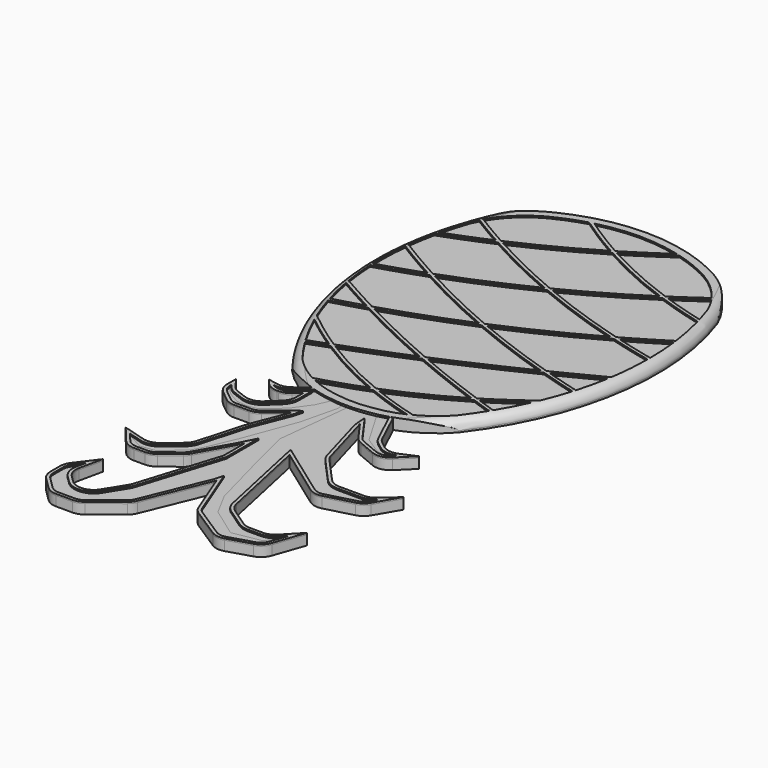
from build123d import *

# Parameters (mm, degrees)
F1_DEPTH    = 3.5
F2_DEPTH    = 3
F3_T2_ANGLE = 85.5642874653
F4_T2_ANGLE = 85.5642874653
F6_DEPTH    = 3.5
F7_DEPTH    = 3
F8_DEPTH    = 3


# Not quite as in the source:
# - a fillet or chamfer that OpenCascade refuses, or shapes differently, is made with other operations: its cross-section is extruded or revolved along the edge and cut away or added


with BuildPart() as f1:
    # F0 (on Top) → F1 (new body)
    with BuildSketch(Plane.XY):
        with BuildLine():
            ThreePointArc((39.7315398477, 36.3386330437), (33.4423121167, 45.7430060507), (24.2254083848, 52.3038979642))
            ThreePointArc((24.2254083848, 52.3038979642), (12.4021780274, 56.4955911336), (-0.0584908148, 57.9415509231))
            ThreePointArc((-0.0584908148, 57.9415509231), (-12.5140877618, 56.4525336617), (-24.3227603276, 52.220002511))
            ThreePointArc((-24.3227603276, 52.220002511), (-33.5169334965, 45.6272946572), (-39.7736206147, 36.2012412195))
            ThreePointArc((-39.7736206147, 36.2012412195), (-43.6986897086, -8.1006975064), (-26.0042863122, -48.904815322))
            ThreePointArc((-26.0042863122, -48.904815322), (-16.9940798529, -55.9254045688), (-6.1260214845, -59.4407709951))
            ThreePointArc((-6.1260214845, -59.4407709951), (0.0009993004, -59.9785797086), (6.1295521331, -59.458520012))
            ThreePointArc((6.1295521331, -59.458520012), (17.1434555414, -55.9337566242), (26.2564282234, -48.8145042671))
            ThreePointArc((26.2564282234, -48.8145042671), (43.8097002393, -7.9494754063), (39.7315398477, 36.3386330437))
        make_face()
        with BuildLine():
            ThreePointArc((-40.0970089943, 26.1242975118), (-38.8944879448, 30.7450005657), (-37.4426184057, 35.2935199323))
            ThreePointArc((-37.4426184057, 35.2935199323), (-36.900501737, 36.4754500531), (-36.3056990744, 37.631762764))
            Line((-36.3056990744, 37.631762764), (-35.8127575622, 38.502842185))
            ThreePointArc((-35.8127575622, 38.502842185), (-31.1708728279, 44.4434367545), (-25.1488920077, 48.9792392994))
            ThreePointArc((-25.1488920077, 48.9792392994), (-24.202818539, 49.4910997693), (-23.2383287957, 49.9673514717))
            ThreePointArc((-23.2383287957, 49.9673514717), (-18.8905512308, 51.8705626769), (-14.3907721795, 53.3796588087))
            Line((-14.3907721795, 53.3796588087), (-13.0000428192, 53.7579055058))
            ThreePointArc((-13.0000428192, 53.7579055058), (-6.5788228993, 54.9973775577), (-0.0541705549, 55.441526197))
            ThreePointArc((-0.0541705549, 55.441526197), (6.4719778709, 55.0199304752), (12.8974432578, 53.8026586115))
            Line((12.8974432578, 53.8026586115), (14.1571575869, 53.4664562649))
            ThreePointArc((14.1571575869, 53.4664562649), (18.7302155896, 51.9601532895), (23.1487688598, 50.0475124063))
            ThreePointArc((23.1487688598, 50.0475124063), (24.1148988463, 49.5745969826), (25.062735738, 49.0660093543))
            ThreePointArc((25.062735738, 49.0660093543), (30.1404172888, 45.4459283737), (34.3219911021, 40.8196689039))
            Line((34.3219911021, 40.8196689039), (34.9078057763, 40.009223861))
            ThreePointArc((34.9078057763, 40.009223861), (34.9011185046, 40.0043902588), (34.8944310771, 39.9995568721))
            ThreePointArc((34.8944310771, 39.9995568721), (36.2527289653, 37.7680473139), (37.4036887939, 35.4228608534))
            ThreePointArc((37.4036887939, 35.4228608534), (38.3055922705, 32.732499506), (39.1201095297, 30.0144053767))
            Line((39.1201095297, 30.0144053767), (39.4251816785, 28.9053924173))
            ThreePointArc((39.4251816785, 28.9053924173), (40.7486142674, 23.2184984056), (41.6912294439, 17.4562320159))
            Line((41.6912294439, 17.4562320159), (41.8265280279, 16.3581858097))
            ThreePointArc((41.8265280279, 16.3581858097), (42.2625598888, 11.4202149898), (42.4192747958, 6.4655081327))
            Line((42.4192747958, 6.4655081327), (42.416776229, 5.4413095421))
            ThreePointArc((42.416776229, 5.4413095421), (42.1205387685, -1.0759263813), (41.3413023404, -7.5531874771))
            Line((41.3413023404, -7.5531874771), (41.1358736734, -8.7942245025))
            ThreePointArc((41.1358736734, -8.7942245025), (40.1573274531, -13.6379002722), (38.907890834, -18.4188683543))
            Line((38.907890834, -18.4188683543), (38.6223423949, -19.3776744647))
            ThreePointArc((38.6223423949, -19.3776744647), (37.1170005182, -23.8866962669), (35.3698823567, -28.3076588214))
            Line((35.3698823567, -28.3076588214), (34.5418820463, -30.1864022845))
            ThreePointArc((34.5418820463, -30.1864022845), (32.2330847183, -34.8863148314), (29.6482784375, -39.4402691065))
            Line((29.6482784375, -39.4402691065), (29.1096093326, -40.3150889597))
            ThreePointArc((29.1096093326, -40.3150889597), (26.8032343681, -43.8225698968), (24.3318836627, -47.2158299358))
            ThreePointArc((24.3318836627, -47.2158299358), (20.411122507, -50.8584456821), (15.9121483231, -53.7567639543))
            Line((15.9121483231, -53.7567639543), (14.5641869359, -54.423573784))
            ThreePointArc((14.5641869359, -54.423573784), (10.2550793614, -56.0398267629), (5.7513142175, -56.9868121434))
            ThreePointArc((5.7513142175, -56.9868121434), (0.0061228743, -57.4785844731), (-5.7376658882, -56.9706925089))
            ThreePointArc((-5.7376658882, -56.9706925089), (-10.1775982453, -56.0167637045), (-14.4257956532, -54.4118343343))
            Line((-14.4257956532, -54.4118343343), (-15.7620953063, -53.7488472631))
            ThreePointArc((-15.7620953063, -53.7488472631), (-20.2051500874, -50.8874144148), (-24.0852785257, -47.2994989983))
            ThreePointArc((-24.0852785257, -47.2994989983), (-26.7226719537, -43.6928037188), (-29.17320975, -39.9566346324))
            Line((-29.17320975, -39.9566346324), (-29.7061139942, -39.0859911492))
            ThreePointArc((-29.7061139942, -39.0859911492), (-32.4866064741, -34.1276140293), (-34.9404764608, -28.9997329677))
            Line((-34.9404764608, -28.9997329677), (-35.7785749676, -27.0270967528))
            ThreePointArc((-35.7785749676, -27.0270967528), (-37.295385716, -23.0621625792), (-38.6188184162, -19.0285607476))
            ThreePointArc((-38.6188184162, -19.0285607476), (-38.629570307, -19.0314780129), (-38.6403223078, -19.0343948724))
            Line((-38.6403223078, -19.0343948724), (-38.9021259101, -18.0692737018))
            ThreePointArc((-38.9021259101, -18.0692737018), (-40.0798201962, -13.5491012604), (-41.0155101079, -8.9727045205))
            Line((-41.0155101079, -8.9727045205), (-41.2316761881, -7.6958807575))
            ThreePointArc((-41.2316761881, -7.6958807575), (-41.8789071815, -2.8369342823), (-42.2540237352, 2.0505555007))
            Line((-42.2540237352, 2.0505555007), (-42.298163194, 3.0808137876))
            ThreePointArc((-42.298163194, 3.0808137876), (-42.3091504015, 9.256209015), (-41.8861332565, 15.4171085783))
            Line((-41.8861332565, 15.4171085783), (-41.7644020186, 16.5189644431))
            ThreePointArc((-41.7644020186, 16.5189644431), (-41.1636895809, 20.7593121742), (-40.356966004, 24.9653318346))
            Line((-40.356966004, 24.9653318346), (-40.0970089943, 26.1242975118))
        make_face(mode=Mode.SUBTRACT)
        with BuildLine():
            ThreePointArc((-26.2523213152, 31.688925786), (-33.1289558692, 28.7928878291), (-40.0970089943, 26.1242975118))
            Line((-40.0970089943, 26.1242975118), (-40.356966004, 24.9653318346))
            Line((-40.356966004, 24.9653318346), (-39.7547528209, 25.1846908325))
            ThreePointArc((-39.7547528209, 25.1846908325), (-32.4057639474, 28.0061467928), (-25.1584979733, 31.0794816427))
            ThreePointArc((-25.1584979733, 31.0794816427), (-13.2812928479, 24.9048932643), (-1.0943151594, 19.366742124))
            ThreePointArc((-1.0943151594, 19.366742124), (-14.0350911684, 13.3472518363), (-27.2922981924, 8.0610046831))
            ThreePointArc((-27.2922981924, 8.0610046831), (-34.5879692857, 12.1879723769), (-41.7644020186, 16.5189644431))
            Line((-41.7644020186, 16.5189644431), (-41.8861332565, 15.4171085783))
            ThreePointArc((-41.8861332565, 15.4171085783), (-35.2647214681, 11.4253075933), (-28.5420835894, 7.6064453114))
            ThreePointArc((-28.5420835894, 7.6064453114), (-35.3879990542, 5.2459846259), (-42.298163194, 3.0808137876))
            Line((-42.298163194, 3.0808137876), (-42.2540237352, 2.0505555007))
            Line((-42.2540237352, 2.0505555007), (-42.0127415165, 2.1224117499))
            ThreePointArc((-42.0127415165, 2.1224117499), (-34.6570110659, 4.4341449671), (-27.3742161903, 6.966294198))
            ThreePointArc((-27.3742161903, 6.966294198), (-14.8173077766, 0.5006160389), (-1.9684375384, -5.3634675696))
            ThreePointArc((-1.9684375384, -5.3634675696), (-14.9184813536, -10.4478909701), (-28.0944629845, -14.9142658081))
            ThreePointArc((-28.0944629845, -14.9142658081), (-34.6981130539, -11.3688511918), (-41.2316761881, -7.6958807575))
            Line((-41.2316761881, -7.6958807575), (-41.0155101079, -8.9727045205))
            ThreePointArc((-41.0155101079, -8.9727045205), (-35.2576995917, -12.2023800976), (-29.4456332141, -15.3333656765))
            ThreePointArc((-29.4456332141, -15.3333656765), (-34.1624327966, -16.7408847084), (-38.9021259101, -18.0692737018))
            Line((-38.9021259101, -18.0692737018), (-38.6403223078, -19.0343948724))
            ThreePointArc((-38.6403223078, -19.0343948724), (-38.629570307, -19.0314780129), (-38.6188184162, -19.0285607476))
            ThreePointArc((-38.6188184162, -19.0285607476), (-33.3913124238, -17.558333374), (-28.1917416686, -15.9921752109))
            ThreePointArc((-28.1917416686, -15.9921752109), (-15.3584122415, -22.4049159564), (-2.2962120371, -28.3375809455))
            ThreePointArc((-2.2962120371, -28.3375809455), (-12.5032813151, -32.5387395342), (-22.7926864891, -36.5340039682))
            ThreePointArc((-22.7926864891, -36.5340039682), (-29.4248776362, -31.970753628), (-35.7785749676, -27.0270967528))
            Line((-35.7785749676, -27.0270967528), (-34.9404764608, -28.9997329677))
            ThreePointArc((-34.9404764608, -28.9997329677), (-29.5459644351, -33.1199351159), (-23.9560126956, -36.9708136244))
            ThreePointArc((-23.9560126956, -36.9708136244), (-26.8281149722, -38.0364175259), (-29.7061139942, -39.0859911492))
            Line((-29.7061139942, -39.0859911492), (-29.17320975, -39.9566346324))
            ThreePointArc((-29.17320975, -39.9566346324), (-26.0385639281, -38.8112749252), (-22.9109202023, -37.6469304693))
            ThreePointArc((-22.9109202023, -37.6469304693), (-12.3569735497, -43.7692550993), (-1.3050479552, -48.9387414834))
            ThreePointArc((-1.3050479552, -48.9387414834), (-8.472559111, -51.5271709824), (-15.7620953063, -53.7488472631))
            Line((-15.7620953063, -53.7488472631), (-14.4257956532, -54.4118343343))
            ThreePointArc((-14.4257956532, -54.4118343343), (-7.1339721558, -52.131639568), (0.0334035434, -49.4861332506))
            ThreePointArc((0.0334035434, -49.4861332506), (7.2303386494, -52.1563198191), (14.5641869359, -54.423573784))
            Line((14.5641869359, -54.423573784), (15.9121483231, -53.7567639543))
            ThreePointArc((15.9121483231, -53.7567639543), (8.5767259151, -51.5531714258), (1.3754196272, -48.9444495771))
            ThreePointArc((1.3754196272, -48.9444495771), (12.2821043467, -43.9679731053), (22.7603812807, -38.1433012572))
            ThreePointArc((22.7603812807, -38.1433012572), (25.9302878911, -39.2429572523), (29.1096093326, -40.3150889597))
            Line((29.1096093326, -40.3150889597), (29.6482784375, -39.4402691065))
            ThreePointArc((29.6482784375, -39.4402691065), (26.7492432711, -38.4658272589), (23.8580200934, -37.4684455132))
            ThreePointArc((23.8580200934, -37.4684455132), (29.2778014505, -33.9416422157), (34.5418820463, -30.1864022845))
            Line((34.5418820463, -30.1864022845), (35.3698823567, -28.3076588214))
            ThreePointArc((35.3698823567, -28.3076588214), (29.1194271433, -32.8384264787), (22.6445025341, -37.0421625844))
            ThreePointArc((22.6445025341, -37.0421625844), (11.3792565478, -32.8655194701), (0.2494566642, -28.3402935766))
            ThreePointArc((0.2494566642, -28.3402935766), (13.7044169839, -22.3617159163), (26.9946569189, -16.0254022787))
            ThreePointArc((26.9946569189, -16.0254022787), (32.7914994599, -17.7605052254), (38.6223423949, -19.3776744647))
            Line((38.6223423949, -19.3776744647), (38.907890834, -18.4188683543))
            ThreePointArc((38.907890834, -18.4188683543), (33.588471101, -16.9490313605), (28.2972499397, -15.3807119709))
            ThreePointArc((28.2972499397, -15.3807119709), (34.7381459321, -12.1295408083), (41.1358736734, -8.7942245025))
            Line((41.1358736734, -8.7942245025), (41.3413023404, -7.5531874771))
            ThreePointArc((41.3413023404, -7.5531874771), (34.1530600722, -11.3057633069), (26.9102193839, -14.9518449059))
            ThreePointArc((26.9102193839, -14.9518449059), (13.6383638025, -10.4669547279), (0.5925078958, -5.3618558902))
            ThreePointArc((0.5925078958, -5.3618558902), (15.0614515903, 1.3227578367), (29.1484304399, 8.7787231801))
            ThreePointArc((29.1484304399, 8.7787231801), (35.6527463944, 7.0474325621), (42.200789062, 5.48966799))
            Line((42.200789062, 5.48966799), (42.416776229, 5.4413095421))
            Line((42.416776229, 5.4413095421), (42.4192747958, 6.4655081327))
            ThreePointArc((42.4192747958, 6.4655081327), (36.3789153207, 7.896211033), (30.37560308, 9.4751649644))
            ThreePointArc((30.37560308, 9.4751649644), (36.1400189189, 12.8518706932), (41.8265280279, 16.3581858097))
            Line((41.8265280279, 16.3581858097), (41.6912294439, 17.4562320159))
            ThreePointArc((41.6912294439, 17.4562320159), (35.4026816436, 13.5755496691), (29.0186311962, 9.8540675988))
            ThreePointArc((29.0186311962, 9.8540675988), (15.0166306719, 14.2497439487), (1.294062841, 19.4525433283))
            ThreePointArc((1.294062841, 19.4525433283), (13.3501967675, 26.0180339732), (25.0371504375, 33.2201966051))
            ThreePointArc((25.0371504375, 33.2201966051), (24.444258116, 33.4297142025), (23.8521848554, 33.6415353124))
            ThreePointArc((23.8521848554, 33.6415353124), (24.3780823357, 33.9840923007), (24.9031353168, 34.3279422928))
            ThreePointArc((24.9031353168, 34.3279422928), (12.8532502016, 39.1576425097), (1.232406082, 44.9439813717))
            ThreePointArc((1.232406082, 44.9439813717), (7.4172624418, 48.8661931101), (13.4730288082, 52.9849170422))
            Line((13.4730288082, 52.9849170422), (14.1571575869, 53.4664562649))
            Line((14.1571575869, 53.4664562649), (12.8974432578, 53.8026586115))
            ThreePointArc((12.8974432578, 53.8026586115), (6.6310497484, 49.5464009998), (0.2262032944, 45.501483402))
            ThreePointArc((0.2262032944, 45.501483402), (-6.4870881422, 49.4692312862), (-13.0000428192, 53.7579055058))
            Line((-13.0000428192, 53.7579055058), (-14.3907721795, 53.3796588087))
            Line((-14.3907721795, 53.3796588087), (-13.5701001421, 52.9363005832))
            ThreePointArc((-13.5701001421, 52.9363005832), (-7.2575152667, 48.7716131717), (-0.7571509133, 44.9065630665))
            ThreePointArc((-0.7571509133, 44.9065630665), (-12.74106826, 38.1828540042), (-25.1096605861, 32.1961635664))
            ThreePointArc((-25.1096605861, 32.1961635664), (-30.5000529705, 35.2835806979), (-35.8127575622, 38.502842185))
            Line((-35.8127575622, 38.502842185), (-36.3056990744, 37.631762764))
            ThreePointArc((-36.3056990744, 37.631762764), (-31.3132830809, 34.6023655231), (-26.2523213152, 31.688925786))
        make_face()
        with BuildLine():
            ThreePointArc((21.5413811084, -37.7122051272), (11.0026239497, -43.4906961277), (0.0357040293, -48.4083203662))
            ThreePointArc((0.0357040293, -48.4083203662), (-11.1028669453, -43.2930928986), (-21.7415261705, -37.2060373469))
            ThreePointArc((-21.7415261705, -37.2060373469), (-11.3408702356, -33.150181056), (-1.0246078322, -28.8842293271))
            ThreePointArc((-1.0246078322, -28.8842293271), (10.1892745774, -33.4748808284), (21.5413811084, -37.7122051272))
        make_face(mode=Mode.SUBTRACT)
        with BuildLine():
            ThreePointArc((25.610448662, -15.592047066), (12.3748643117, -21.8719878559), (-1.0234472948, -27.7968165887))
            ThreePointArc((-1.0234472948, -27.7968165887), (-14.0457162076, -21.9215329651), (-26.8416467865, -15.5683758039))
            ThreePointArc((-26.8416467865, -15.5683758039), (-13.6504815899, -11.0473270966), (-0.6875902156, -5.9082447005))
            ThreePointArc((-0.6875902156, -5.9082447005), (12.3476508262, -11.0591307834), (25.610448662, -15.592047066))
        make_face(mode=Mode.SUBTRACT)
        with BuildLine():
            ThreePointArc((0.2479479948, 44.345023142), (11.8353254417, 38.5197142438), (23.8521848554, 33.6415353124))
            ThreePointArc((23.8521848554, 33.6415353124), (12.150254978, 26.4796674086), (0.0801672264, 19.9573598111))
            ThreePointArc((0.0801672264, 19.9573598111), (-12.122388639, 25.45440003), (-24.0161032078, 31.5911234694))
            ThreePointArc((-24.0161032078, 31.5911234694), (-11.692337092, 37.6032906289), (0.2479479948, 44.345023142))
        make_face(mode=Mode.SUBTRACT)
        with BuildLine():
            ThreePointArc((-0.6882739483, -4.8220095942), (-13.5520247939, 0.999684532), (-26.1248663789, 7.4255590093))
            ThreePointArc((-26.1248663789, 7.4255590093), (-12.8427171877, 12.7742778018), (0.1196950161, 18.8570526387))
            ThreePointArc((0.1196950161, 18.8570526387), (13.8152948172, 13.6092128203), (27.7918103061, 9.1632830568))
            ThreePointArc((27.7918103061, 9.1632830568), (13.7404821908, 1.7863336572), (-0.6882739483, -4.8220095942))
        make_face(mode=Mode.SUBTRACT)
        with BuildLine():
            ThreePointArc((34.3219911021, 40.8196689039), (29.6489606376, 37.5209965158), (24.9031353168, 34.3279422928))
            ThreePointArc((24.9031353168, 34.3279422928), (25.4961146486, 34.118947077), (26.0899069289, 33.9122728984))
            ThreePointArc((26.0899069289, 33.9122728984), (30.5239796689, 36.9099045828), (34.8944310771, 39.9995568721))
            ThreePointArc((34.8944310771, 39.9995568721), (34.9011185046, 40.0043902588), (34.9078057763, 40.009223861))
            Line((34.9078057763, 40.009223861), (34.3219911021, 40.8196689039))
        make_face()
        with BuildLine():
            ThreePointArc((26.0899069289, 33.9122728984), (25.4961146486, 34.118947077), (24.9031353168, 34.3279422928))
            ThreePointArc((24.9031353168, 34.3279422928), (24.3780823357, 33.9840923007), (23.8521848554, 33.6415353124))
            ThreePointArc((23.8521848554, 33.6415353124), (24.444258116, 33.4297142025), (25.0371504375, 33.2201966051))
            ThreePointArc((25.0371504375, 33.2201966051), (25.5639543178, 33.5655872948), (26.0899069289, 33.9122728984))
        make_face()
        with BuildLine():
            ThreePointArc((39.1201095297, 30.0144053767), (32.5637631454, 31.8254607214), (26.0899069289, 33.9122728984))
            ThreePointArc((26.0899069289, 33.9122728984), (25.5639543178, 33.5655872948), (25.0371504375, 33.2201966051))
            ThreePointArc((25.0371504375, 33.2201966051), (31.9090676633, 30.9779995191), (38.8743055461, 29.0450858207))
            Line((38.8743055461, 29.0450858207), (39.4251816785, 28.9053924173))
            Line((39.4251816785, 28.9053924173), (39.1201095297, 30.0144053767))
        make_face()
    extrude(amount=F1_DEPTH)

    # F3: fillet of radius 3 on 1 edges, made by hand

    # F3_s1 → F3_t2 (revolve, cut)
    with BuildSketch(Plane(origin=(-25.0202878659, -19.7071440351, 0), x_dir=(0, 0, 1), z_dir=(-0.785580343, -0.6187596663, 0))):
        with BuildLine():
            ThreePointArc((0.5, -57.3830921814), (2.6213203436, -56.504412525), (3.5, -54.3830921814))
            Line((3.5, -54.3830921814), (3.5, -57.3830921814))
            Line((3.5, -57.3830921814), (0.5, -57.3830921814))
        make_face()
    revolve(axis=Axis((-45.400476836, 6.1676450203, 3.5), (0, 0, 1)), revolution_arc=F3_T2_ANGLE, mode=Mode.SUBTRACT)

    # F4: fillet of radius 3 on 1 edges, made by hand

    # F4_s1 → F4_t2 (revolve, cut)
    with BuildSketch(Plane(origin=(16.8313827916, 25.341059687, 0), x_dir=(0, 0, 1), z_dir=(0.5532734825, 0.832999672, 0))):
        with BuildLine():
            ThreePointArc((0.5, -55.949558136), (2.6213203436, -55.0708784796), (3.5, -52.949558136))
            Line((3.5, -52.949558136), (3.5, -55.949558136))
            Line((3.5, -55.949558136), (0.5, -55.949558136))
        make_face()
    revolve(axis=Axis((45.4621634791, 6.3246635564, 3.5), (0, 0, 1)), revolution_arc=F4_T2_ANGLE, mode=Mode.SUBTRACT)

    # F5 (on Top) → F6 (join)
    with BuildSketch(Plane.XY):
        with BuildLine():
            ThreePointArc((-11.2406425351, -58.1860276718), (-11.85513961, -57.9802448121), (-12.4660098375, -57.763932987))
            Line((-12.4660098375, -57.763932987), (-16.5981199184, -60.8148670105))
            ThreePointArc((-16.5981199184, -60.8148670105), (-18.4560293791, -61.6672572751), (-20.4997954923, -61.7048976981))
            Line((-20.4997954923, -61.7048976981), (-23.6099157482, -61.1149892211))
            Line((-23.6099157482, -61.1149892211), (-22.204564583, -62.7466937757))
            ThreePointArc((-22.204564583, -62.7466937757), (-20.4999125979, -64.0287614999), (-18.416033223, -64.4837151141))
            Line((-18.416033223, -64.4837151141), (-17.8405212143, -64.4837151141))
            ThreePointArc((-17.8405212143, -64.4837151141), (-16.1139213921, -64.1761401785), (-14.5997451063, -63.291256309))
            Line((-14.5997451063, -63.291256309), (-12.4660098375, -61.4751345314))
            Line((-12.4660098375, -61.4751345314), (-12.4660098375, -64.2680988657))
            ThreePointArc((-12.4660098375, -64.2680988657), (-12.8778616237, -66.2552817653), (-14.0455682234, -67.9150947269))
            Line((-14.0455682234, -67.9150947269), (-17.2625708293, -70.9322545059))
            ThreePointArc((-17.2625708293, -70.9322545059), (-19.709137439, -72.1894982979), (-22.4504511986, -71.9624542504))
            Line((-22.4504511986, -71.9624542504), (-25.4652231505, -70.8232192104))
            ThreePointArc((-25.4652231505, -70.8232192104), (-26.7189408477, -70.1300682703), (-27.7246498228, -69.109864493))
            Line((-27.7246498228, -69.109864493), (-30.0487410277, -65.9522041678))
            Line((-30.0487410277, -65.9522041678), (-30.0487410277, -69.4568890433))
            ThreePointArc((-30.0487410277, -69.4568890433), (-29.564074372, -71.6043910064), (-28.204035114, -73.3355639223))
            Line((-28.204035114, -73.3355639223), (-25.0261640417, -75.9207554527))
            ThreePointArc((-25.0261640417, -75.9207554527), (-23.5451796146, -76.7534165225), (-21.8708700672, -77.042080462))
            Line((-21.8708700672, -77.042080462), (-17.1831318895, -77.042080462))
            ThreePointArc((-17.1831318895, -77.042080462), (-15.5230418259, -76.7584456851), (-14.0512954765, -75.9397208297))
            Line((-14.0512954765, -75.9397208297), (-8.185690443, -71.2265830792))
            Line((-8.185690443, -71.2265830792), (-12.7783518406, -82.8575778448))
            Line((-12.7783518406, -82.8575778448), (-17.0428670856, -97.8528116547))
            ThreePointArc((-17.0428670856, -97.8528116547), (-17.6604376583, -99.2107875146), (-18.6511543341, -100.3261225838))
            Line((-18.6511543341, -100.3261225838), (-23.2902932274, -104.192250631))
            ThreePointArc((-23.2902932274, -104.192250631), (-25.4627560322, -105.2442827816), (-27.8749264104, -105.1559631869))
            Line((-27.8749264104, -105.1559631869), (-35.1496301591, -103.0610650778))
            Line((-35.1496301591, -103.0610650778), (-30.5810507571, -108.5377954723))
            ThreePointArc((-30.5810507571, -108.5377954723), (-28.8611898085, -109.8634318077), (-26.7415438219, -110.3349551558))
            Line((-26.7415438219, -110.3349551558), (-23.2923726828, -110.3349551558))
            ThreePointArc((-23.2923726828, -110.3349551558), (-21.6658484321, -110.0630011371), (-20.2162601079, -109.2767226769))
            Line((-20.2162601079, -109.2767226769), (-15.1005370927, -105.2844678676))
            ThreePointArc((-15.1005370927, -105.2844678676), (-14.3838703522, -104.6007403517), (-13.8160466204, -103.7891550249))
            Line((-13.8160466204, -103.7891550249), (-6.9706922621, -91.5878767008))
            Line((-6.9706922621, -91.5878767008), (-6.9706922621, -99.7316465933))
            Line((-6.9706922621, -99.7316465933), (-14.9715564629, -125.3131624998))
            ThreePointArc((-14.9715564629, -125.3131624998), (-15.1970540612, -125.9012569659), (-15.4946970845, -126.4563361482))
            Line((-15.4946970845, -126.4563361482), (-19.3489654972, -132.6697018922))
            ThreePointArc((-19.3489654972, -132.6697018922), (-21.1666567483, -134.403142811), (-23.5978718614, -135.0340247154))
            Line((-23.5978718614, -135.0340247154), (-23.749616452, -135.0340247154))
            ThreePointArc((-23.749616452, -135.0340247154), (-25.6316256802, -134.6663072179), (-27.2368158127, -133.6172411897))
            Line((-27.2368158127, -133.6172411897), (-29.1772149061, -131.7288376458))
            ThreePointArc((-29.1772149061, -131.7288376458), (-30.4788518976, -129.5833435351), (-30.5741993785, -127.0756927031))
            Line((-30.5741993785, -127.0756927031), (-28.9786346257, -119.7919994593))
            Line((-28.9786346257, -119.7919994593), (-33.8844086411, -126.2815765127))
            ThreePointArc((-33.8844086411, -126.2815765127), (-34.6362301506, -127.7065982361), (-34.8958224058, -129.2967348199))
            Line((-34.8958224058, -129.2967348199), (-34.8958224058, -132.954178789))
            ThreePointArc((-34.8958224058, -132.954178789), (-34.5082344999, -134.8843742682), (-33.4055605373, -136.5153215712))
            Line((-33.4055605373, -136.5153215712), (-29.9196178603, -139.9509449922))
            ThreePointArc((-29.9196178603, -139.9509449922), (-28.3064933185, -141.0161243127), (-26.4098798405, -141.3898020983))
            Line((-26.4098798405, -141.3898020983), (-21.271502647, -141.3898020983))
            ThreePointArc((-21.271502647, -141.3898020983), (-19.6200858194, -141.1092112137), (-18.1540179993, -140.2989310586))
            Line((-18.1540179993, -140.2989310586), (-9.9490926932, -133.7555988565))
            ThreePointArc((-9.9490926932, -133.7555988565), (-9.0674898945, -132.8476861746), (-8.4420732772, -131.7475121032))
            Line((-8.4420732772, -131.7475121032), (0, -111.2111955881))
            Line((0, -111.2111955881), (5.4608781402, -125.1309921592))
            ThreePointArc((5.4608781402, -125.1309921592), (6.243771637, -126.4687481633), (7.3987404493, -127.5024601137))
            Line((7.3987404493, -127.5024601137), (16.6539848106, -133.4927262236))
            ThreePointArc((16.6539848106, -133.4927262236), (18.6785947288, -134.2470629419), (20.8324450105, -134.0767744541))
            Line((20.8324450105, -134.0767744541), (28.1438036059, -131.8417340671))
            ThreePointArc((28.1438036059, -131.8417340671), (30.1488939439, -130.6631283876), (31.4038405112, -128.7049129438))
            Line((31.4038405112, -128.7049129438), (34.7734875977, -119.0313622355))
            Line((34.7734875977, -119.0313622355), (29.7843459334, -124.2219127935))
            ThreePointArc((29.7843459334, -124.2219127935), (28.1385808212, -125.3572544369), (26.1795657861, -125.757008791))
            Line((26.1795657861, -125.757008791), (22.2305893073, -125.757008791))
            ThreePointArc((22.2305893073, -125.757008791), (20.7554772225, -125.534460443), (19.4116786437, -124.8866265064))
            Line((19.4116786437, -124.8866265064), (13.6600243431, -120.9605003618))
            ThreePointArc((13.6600243431, -120.9605003618), (12.328677467, -119.6193162316), (11.5901964634, -117.879803316))
            Line((11.5901964634, -117.879803316), (5.4574797355, -89.2968487582))
            Line((5.4574797355, -89.2968487582), (21.1351129427, -100.5775695251))
            ThreePointArc((21.1351129427, -100.5775695251), (23.1493256255, -101.4362324219), (25.3373024997, -101.3519003414))
            Line((25.3373024997, -101.3519003414), (34.0518879685, -99.0404156757))
            ThreePointArc((34.0518879685, -99.0404156757), (35.7997585425, -98.185038548), (37.0887147929, -96.7271930971))
            Line((37.0887147929, -96.7271930971), (41.3617279304, -89.4032176392))
            Line((41.3617279304, -89.4032176392), (36.6451902439, -93.5975401487))
            ThreePointArc((36.6451902439, -93.5975401487), (35.0999680917, -94.5346336132), (33.3225549366, -94.8612191866))
            Line((33.3225549366, -94.8612191866), (25.6929397614, -94.8612191866))
            ThreePointArc((25.6929397614, -94.8612191866), (23.6665003866, -94.4321647523), (21.9878421394, -93.218636534))
            Line((21.9878421394, -93.218636534), (14.8472454835, -85.338588916))
            ThreePointArc((14.8472454835, -85.338588916), (14.1802948274, -84.407113299), (13.7428714702, -83.3482786522))
            Line((13.7428714702, -83.3482786522), (8.7073437039, -65.6333313506))
            Line((8.7073437039, -65.6333313506), (12.9932515446, -71.6159779104))
            ThreePointArc((12.9932515446, -71.6159779104), (13.9437349098, -72.6159244887), (15.1313050546, -73.3180561987))
            Line((15.1313050546, -73.3180561987), (20.7032531396, -75.6446450353))
            ThreePointArc((20.7032531396, -75.6446450353), (23.5794447514, -75.9397077469), (26.1380985171, -74.5932935839))
            Line((26.1380985171, -74.5932935839), (30.8116656072, -69.9909566185))
            Line((30.8116656072, -69.9909566185), (26.0912624704, -72.0387569836))
            ThreePointArc((26.0912624704, -72.0387569836), (23.494063184, -72.4147751312), (21.0641552696, -71.423623625))
            Line((21.0641552696, -71.423623625), (19.3320822542, -70.0991356473))
            ThreePointArc((19.3320822542, -70.0991356473), (18.4757346728, -69.2642334686), (17.8421589075, -68.249849627))
            Line((17.8421589075, -68.249849627), (12.9824430528, -57.8846974853))
            ThreePointArc((12.9824430528, -57.8846974853), (12.5077523651, -58.0487608115), (12.0309187906, -58.2064876836))
            ThreePointArc((12.0309187906, -58.2064876836), (12.0300247007, -58.2067768272), (12.0291306036, -58.2070659485))
            Line((12.0291306036, -58.2070659485), (12.0770193952, -58.3092066139))
            Line((12.0770193952, -58.3092066139), (16.9367352499, -68.6743587557))
            ThreePointArc((16.9367352499, -68.6743587557), (17.6970261711, -69.8916193701), (18.7246432726, -70.8935019883))
            Line((18.7246432726, -70.8935019883), (20.456716288, -72.217989966))
            ThreePointArc((20.456716288, -72.217989966), (23.267422595, -73.3935563563), (26.2931438297, -73.0371334441))
            Line((26.2931438297, -73.0371334441), (25.436442331, -73.8807779023))
            ThreePointArc((25.436442331, -73.8807779023), (23.3895193298, -74.9579092267), (21.0885660533, -74.7218590587))
            Line((21.0885660533, -74.7218590587), (15.5166179683, -72.3952702221))
            ThreePointArc((15.5166179683, -72.3952702221), (14.5665618578, -71.8335648573), (13.8061751698, -71.0336075991))
            Line((13.8061751698, -71.0336075991), (10.0482091268, -65.7879085652))
            Line((10.0482091268, -65.7879085652), (7.6262057077, -62.4070634884))
            Line((7.6262057077, -62.4070634884), (7.9396267093, -66.2418748066))
            ThreePointArc((7.9396267093, -66.2418748066), (8.0031206329, -66.7260322671), (8.1135384817, -67.201687419))
            Line((8.1135384817, -67.201687419), (12.7809771217, -83.6217000527))
            ThreePointArc((12.7809771217, -83.6217000527), (13.3058851523, -84.8923016336), (14.1062259425, -86.0100723781))
            Line((14.1062259425, -86.0100723781), (21.2468225984, -93.8901199961))
            ThreePointArc((21.2468225984, -93.8901199961), (23.2612125026, -95.3463538635), (25.6929397614, -95.8612191866))
            Line((25.6929397614, -95.8612191866), (33.3225549366, -95.8612191866))
            ThreePointArc((33.3225549366, -95.8612191866), (34.9572937771, -95.6342278366), (36.4683420898, -94.9704288112))
            Line((36.4683420898, -94.9704288112), (37.3331243775, -94.3238789783))
            Line((37.3331243775, -94.3238789783), (36.2249715224, -96.2232609959))
            ThreePointArc((36.2249715224, -96.2232609959), (35.1938065278, -97.38953735), (33.7955100765, -98.0738390483))
            Line((33.7955100765, -98.0738390483), (25.0809246077, -100.3853237141))
            ThreePointArc((25.0809246077, -100.3853237141), (23.3305431181, -100.4527893781), (21.7191729809, -99.7658590645))
            Line((21.7191729809, -99.7658590645), (6.0415397737, -88.4851382977))
            Line((6.0415397737, -88.4851382977), (4.0325531736, -87.009049952))
            Line((4.0325531736, -87.009049952), (4.479732005, -89.5066328745))
            Line((4.479732005, -89.5066328745), (10.6124487328, -118.0895874323))
            ThreePointArc((10.6124487328, -118.0895874323), (11.4986259405, -120.1770029387), (13.0962421978, -121.786423901))
            Line((13.0962421978, -121.786423901), (18.8478964984, -125.7125500457))
            ThreePointArc((18.8478964984, -125.7125500457), (20.460454799, -126.4899507724), (22.2305893073, -126.757008791))
            Line((22.2305893073, -126.757008791), (26.1795657861, -126.757008791))
            ThreePointArc((26.1795657861, -126.757008791), (28.530383837, -126.2773035643), (30.5053019789, -124.9148935871))
            Line((30.5053019789, -124.9148935871), (32.3243162103, -123.0224467558))
            Line((32.3243162103, -123.0224467558), (30.4594932602, -128.3759626897))
            ThreePointArc((30.4594932602, -128.3759626897), (29.455536012, -129.9425350361), (27.8514637506, -130.8854195744))
            Line((27.8514637506, -130.8854195744), (20.5401051552, -133.1204599614))
            ThreePointArc((20.5401051552, -133.1204599614), (18.8170249394, -133.2566907508), (17.197337014, -132.6532213796))
            Line((17.197337014, -132.6532213796), (7.9420926526, -126.6629552696))
            ThreePointArc((7.9420926526, -126.6629552696), (7.018117608, -125.835985714), (6.3918028141, -124.7657809167))
            Line((6.3918028141, -124.7657809167), (0.9309246738, -110.8459843456))
            Line((0.9309246738, -110.8459843456), (-0.1832797938, -108.0058734459))
            Line((-0.1832797938, -108.0058734459), (-0.9249008334, -110.8309871606))
            Line((-0.9249008334, -110.8309871606), (-9.3669741106, -131.3673036756))
            ThreePointArc((-9.3669741106, -131.3673036756), (-9.8673074016, -132.2474429279), (-10.5725896367, -132.9737730693))
            Line((-10.5725896367, -132.9737730693), (-18.7775149428, -139.5171052714))
            ThreePointArc((-18.7775149428, -139.5171052714), (-19.9503691923, -140.1653293919), (-21.271502647, -140.3898020983))
            Line((-21.271502647, -140.3898020983), (-26.4098798405, -140.3898020983))
            ThreePointArc((-26.4098798405, -140.3898020983), (-27.9271706144, -140.0908598715), (-29.2176702406, -139.2387164199))
            Line((-29.2176702406, -139.2387164199), (-32.7036129177, -135.8030929988))
            ThreePointArc((-32.7036129177, -135.8030929988), (-33.5857520828, -134.4983351637), (-33.8958224058, -132.954178789))
            Line((-33.8958224058, -132.954178789), (-33.8958224058, -129.2967348199))
            ThreePointArc((-33.8958224058, -129.2967348199), (-33.6881486028, -128.0246255599), (-33.0866913986, -126.8846081876))
            Line((-33.0866913986, -126.8846081876), (-30.9315237787, -124.0336561689))
            Line((-30.9315237787, -124.0336561689), (-31.5510361669, -126.8617069823))
            ThreePointArc((-31.5510361669, -126.8617069823), (-31.4366191895, -129.8708879919), (-29.8746547938, -132.4454809343))
            Line((-29.8746547938, -132.4454809343), (-27.9342557005, -134.3338844783))
            ThreePointArc((-27.9342557005, -134.3338844783), (-26.0080275343, -135.5927637168), (-23.749616452, -136.0340247154))
            Line((-23.749616452, -136.0340247154), (-23.5978718614, -136.0340247154))
            ThreePointArc((-23.5978718614, -136.0340247154), (-20.6804137148, -135.2769664273), (-18.4991842054, -133.196837317))
            Line((-18.4991842054, -133.196837317), (-14.6449157927, -126.983471573))
            ThreePointArc((-14.6449157927, -126.983471573), (-14.2877441634, -126.3173765518), (-14.0171470445, -125.6116631898))
            Line((-14.0171470445, -125.6116631898), (-5.9706922621, -99.8843785067))
            Line((-5.9706922621, -99.8843785067), (-5.9706922621, -93.2434648275))
            Line((-5.9706922621, -93.2434648275), (-5.9706922621, -87.2892588377))
            Line((-5.9706922621, -87.2892588377), (-8.6178081697, -92.4799508016))
            Line((-8.6178081697, -92.4799508016), (-14.6881672493, -103.2998641007))
            ThreePointArc((-14.6881672493, -103.2998641007), (-15.1424262322, -103.9491323584), (-15.7157596215, -104.4961143681))
            Line((-15.7157596215, -104.4961143681), (-20.8314826367, -108.4883691774))
            ThreePointArc((-20.8314826367, -108.4883691774), (-21.9911532895, -109.1173919421), (-23.2923726828, -109.3349551558))
            Line((-23.2923726828, -109.3349551558), (-26.7415438219, -109.3349551558))
            ThreePointArc((-26.7415438219, -109.3349551558), (-28.4372606017, -108.9577364794), (-29.8131493529, -107.8972274171))
            Line((-29.8131493529, -107.8972274171), (-32.2931098555, -104.9242956003))
            Line((-32.2931098555, -104.9242956003), (-28.1516511779, -106.1169124067))
            ThreePointArc((-28.1516511779, -106.1169124067), (-25.2570467133, -106.2228959208), (-22.6500913378, -104.9604573353))
            Line((-22.6500913378, -104.9604573353), (-18.0109524445, -101.0943292881))
            ThreePointArc((-18.0109524445, -101.0943292881), (-16.8220924291, -99.7559272001), (-16.0810077391, -98.1263561622))
            Line((-16.0810077391, -98.1263561622), (-11.8300433066, -83.1787708163))
            Line((-11.8300433066, -83.1787708163), (-7.2540071059, -71.5898796507))
            Line((-7.2540071059, -71.5898796507), (-6.5818647854, -68.9077302814))
            Line((-6.5818647854, -68.9077302814), (-8.8091650435, -70.4447306681))
            Line((-8.8091650435, -70.4447306681), (-14.6776627731, -75.1601927611))
            ThreePointArc((-14.6776627731, -75.1601927611), (-15.855059846, -75.8151726417), (-17.1831318895, -76.042080462))
            Line((-17.1831318895, -76.042080462), (-21.8708700672, -76.042080462))
            ThreePointArc((-21.8708700672, -76.042080462), (-23.2103176976, -75.8111493117), (-24.3951052327, -75.1450204596))
            Line((-24.3951052327, -75.1450204596), (-27.572976305, -72.5598289292))
            ThreePointArc((-27.572976305, -72.5598289292), (-28.6610077053, -71.1748906042), (-29.0487410277, -69.4568890433))
            Line((-29.0487410277, -69.4568890433), (-29.0487410277, -68.9978688198))
            Line((-29.0487410277, -68.9978688198), (-28.5300229487, -69.7026326839))
            ThreePointArc((-28.5300229487, -69.7026326839), (-27.323172174, -70.9268772212), (-25.8187109318, -71.7586583524))
            Line((-25.8187109318, -71.7586583524), (-22.8039389799, -72.8978933924))
            ThreePointArc((-22.8039389799, -72.8978933924), (-19.5143624561, -73.1703462504), (-16.5784825135, -71.6616536944))
            Line((-16.5784825135, -71.6616536944), (-13.3614799076, -68.6444939154))
            ThreePointArc((-13.3614799076, -68.6444939154), (-11.9602319828, -66.6527183541), (-11.4660098375, -64.2680988657))
            Line((-11.4660098375, -64.2680988657), (-11.4660098375, -61.4734220935))
            Line((-11.4660098375, -61.4734220935), (-11.4660098375, -59.1814741492))
            Line((-11.4660098375, -59.1814741492), (-13.1141650736, -60.7136262978))
            Line((-13.1141650736, -60.7136262978), (-15.2479003424, -62.5297480753))
            ThreePointArc((-15.2479003424, -62.5297480753), (-16.4592413643, -63.237655167), (-17.8405212143, -63.4837151141))
            Line((-17.8405212143, -63.4837151141), (-18.416033223, -63.4837151141))
            ThreePointArc((-18.416033223, -63.4837151141), (-19.7028554822, -63.2710741446), (-20.8528621711, -62.6557593276))
            Line((-20.8528621711, -62.6557593276), (-20.6861468549, -62.6873808632))
            ThreePointArc((-20.6861468549, -62.6873808632), (-18.2336275099, -62.6422123553), (-16.0041361488, -61.619344034))
            Line((-16.0041361488, -61.619344034), (-11.8720260679, -58.5684100106))
            Line((-11.8720260679, -58.5684100106), (-11.2406425351, -58.1860276718))
        make_face()
    extrude(amount=F6_DEPTH)


with BuildPart() as f2:
    # F0 (on Top) → F2 (new body)
    with BuildSketch(Plane.XY):
        with BuildLine():
            ThreePointArc((-25.1488920077, 48.9792392994), (-31.1708728279, 44.4434367545), (-35.8127575622, 38.502842185))
            ThreePointArc((-35.8127575622, 38.502842185), (-30.5000529705, 35.2835806979), (-25.1096605861, 32.1961635664))
            ThreePointArc((-25.1096605861, 32.1961635664), (-12.74106826, 38.1828540042), (-0.7571509133, 44.9065630665))
            ThreePointArc((-0.7571509133, 44.9065630665), (-7.2575152667, 48.7716131717), (-13.5701001421, 52.9363005832))
            Line((-13.5701001421, 52.9363005832), (-14.3907721795, 53.3796588087))
            ThreePointArc((-14.3907721795, 53.3796588087), (-18.8905512308, 51.8705626769), (-23.2383287957, 49.9673514717))
            ThreePointArc((-23.2383287957, 49.9673514717), (-24.1985929943, 49.4829294721), (-25.1488920077, 48.9792392994))
        make_face()
    extrude(amount=F2_DEPTH)


with BuildPart() as f2b:
    # F0 (on Top) → F2, piece 2 (new body)
    with BuildSketch(Plane.XY):
        with BuildLine():
            ThreePointArc((-0.0541705549, 55.441526197), (-6.5788228993, 54.9973775577), (-13.0000428192, 53.7579055058))
            ThreePointArc((-13.0000428192, 53.7579055058), (-6.4870881422, 49.4692312862), (0.2262032944, 45.501483402))
            ThreePointArc((0.2262032944, 45.501483402), (6.6310497484, 49.5464009998), (12.8974432578, 53.8026586115))
            ThreePointArc((12.8974432578, 53.8026586115), (6.4719778709, 55.0199304752), (-0.0541705549, 55.441526197))
        make_face()
    extrude(amount=F2_DEPTH)


with BuildPart() as f2c:
    # F0 (on Top) → F2, piece 3 (new body)
    with BuildSketch(Plane.XY):
        with BuildLine():
            ThreePointArc((23.1487688598, 50.0475124063), (18.7302155896, 51.9601532895), (14.1571575869, 53.4664562649))
            Line((14.1571575869, 53.4664562649), (13.4730288082, 52.9849170422))
            ThreePointArc((13.4730288082, 52.9849170422), (7.4172624418, 48.8661931101), (1.232406082, 44.9439813717))
            ThreePointArc((1.232406082, 44.9439813717), (12.8532502016, 39.1576425097), (24.9031353168, 34.3279422928))
            ThreePointArc((24.9031353168, 34.3279422928), (29.6489606376, 37.5209965158), (34.3219911021, 40.8196689039))
            ThreePointArc((34.3219911021, 40.8196689039), (30.1404172888, 45.4459283737), (25.062735738, 49.0660093543))
            ThreePointArc((25.062735738, 49.0660093543), (24.1107015648, 49.5664121299), (23.1487688598, 50.0475124063))
        make_face()
    extrude(amount=F2_DEPTH)


with BuildPart() as f2d:
    # F0 (on Top) → F2, piece 4 (new body)
    with BuildSketch(Plane.XY):
        with BuildLine():
            ThreePointArc((0.0801672264, 19.9573598111), (12.150254978, 26.4796674086), (23.8521848554, 33.6415353124))
            ThreePointArc((23.8521848554, 33.6415353124), (11.8353254417, 38.5197142438), (0.2479479948, 44.345023142))
            ThreePointArc((0.2479479948, 44.345023142), (-11.692337092, 37.6032906289), (-24.0161032078, 31.5911234694))
            ThreePointArc((-24.0161032078, 31.5911234694), (-12.122388639, 25.45440003), (0.0801672264, 19.9573598111))
        make_face()
    extrude(amount=F2_DEPTH)


with BuildPart() as f2e:
    # F0 (on Top) → F2, piece 5 (new body)
    with BuildSketch(Plane.XY):
        with BuildLine():
            ThreePointArc((38.8743055461, 29.0450858207), (31.9090676633, 30.9779995191), (25.0371504375, 33.2201966051))
            ThreePointArc((25.0371504375, 33.2201966051), (13.3501967675, 26.0180339732), (1.294062841, 19.4525433283))
            ThreePointArc((1.294062841, 19.4525433283), (15.0166306719, 14.2497439487), (29.0186311962, 9.8540675988))
            ThreePointArc((29.0186311962, 9.8540675988), (35.4026816436, 13.5755496691), (41.6912294439, 17.4562320159))
            ThreePointArc((41.6912294439, 17.4562320159), (40.7486142674, 23.2184984056), (39.4251816785, 28.9053924173))
            Line((39.4251816785, 28.9053924173), (38.8743055461, 29.0450858207))
        make_face()
    extrude(amount=F2_DEPTH)


with BuildPart() as f2f:
    # F0 (on Top) → F2, piece 6 (new body)
    with BuildSketch(Plane.XY):
        with BuildLine():
            ThreePointArc((34.8944310771, 39.9995568721), (30.5239796689, 36.9099045828), (26.0899069289, 33.9122728984))
            ThreePointArc((26.0899069289, 33.9122728984), (32.5637631454, 31.8254607214), (39.1201095297, 30.0144053767))
            ThreePointArc((39.1201095297, 30.0144053767), (38.3055922705, 32.732499506), (37.4036887939, 35.4228608534))
            ThreePointArc((37.4036887939, 35.4228608534), (36.2527289653, 37.7680473139), (34.8944310771, 39.9995568721))
        make_face()
    extrude(amount=F2_DEPTH)


with BuildPart() as f2g:
    # F0 (on Top) → F2, piece 7 (new body)
    with BuildSketch(Plane.XY):
        with BuildLine():
            ThreePointArc((-36.3056990744, 37.631762764), (-36.900501737, 36.4754500531), (-37.4426184057, 35.2935199323))
            ThreePointArc((-37.4426184057, 35.2935199323), (-38.8944879448, 30.7450005657), (-40.0970089943, 26.1242975118))
            ThreePointArc((-40.0970089943, 26.1242975118), (-33.1289558692, 28.7928878291), (-26.2523213152, 31.688925786))
            ThreePointArc((-26.2523213152, 31.688925786), (-31.3132830809, 34.6023655231), (-36.3056990744, 37.631762764))
        make_face()
    extrude(amount=F2_DEPTH)


with BuildPart() as f2h:
    # F0 (on Top) → F2, piece 8 (new body)
    with BuildSketch(Plane.XY):
        with BuildLine():
            ThreePointArc((-28.5420835894, 7.6064453114), (-35.2647214681, 11.4253075933), (-41.8861332565, 15.4171085783))
            ThreePointArc((-41.8861332565, 15.4171085783), (-42.3091504015, 9.256209015), (-42.298163194, 3.0808137876))
            ThreePointArc((-42.298163194, 3.0808137876), (-35.3879990542, 5.2459846259), (-28.5420835894, 7.6064453114))
        make_face()
    extrude(amount=F2_DEPTH)


with BuildPart() as f2i:
    # F0 (on Top) → F2, piece 9 (new body)
    with BuildSketch(Plane.XY):
        with BuildLine():
            Line((-42.0127415165, 2.1224117499), (-42.2540237352, 2.0505555007))
            ThreePointArc((-42.2540237352, 2.0505555007), (-41.8789071815, -2.8369342823), (-41.2316761881, -7.6958807575))
            ThreePointArc((-41.2316761881, -7.6958807575), (-34.6981130539, -11.3688511918), (-28.0944629845, -14.9142658081))
            ThreePointArc((-28.0944629845, -14.9142658081), (-14.9184813536, -10.4478909701), (-1.9684375384, -5.3634675696))
            ThreePointArc((-1.9684375384, -5.3634675696), (-14.8173077766, 0.5006160389), (-27.3742161903, 6.966294198))
            ThreePointArc((-27.3742161903, 6.966294198), (-34.6570110659, 4.4341449671), (-42.0127415165, 2.1224117499))
        make_face()
    extrude(amount=F2_DEPTH)


with BuildPart() as f2j:
    # F0 (on Top) → F2, piece 10 (new body)
    with BuildSketch(Plane.XY):
        with BuildLine():
            ThreePointArc((-29.4456332141, -15.3333656765), (-35.2576995917, -12.2023800976), (-41.0155101079, -8.9727045205))
            ThreePointArc((-41.0155101079, -8.9727045205), (-40.0798201962, -13.5491012604), (-38.9021259101, -18.0692737018))
            ThreePointArc((-38.9021259101, -18.0692737018), (-34.1624327966, -16.7408847084), (-29.4456332141, -15.3333656765))
        make_face()
    extrude(amount=F2_DEPTH)


with BuildPart() as f2k:
    # F0 (on Top) → F2, piece 11 (new body)
    with BuildSketch(Plane.XY):
        with BuildLine():
            ThreePointArc((-28.1917416686, -15.9921752109), (-33.3913124238, -17.558333374), (-38.6188184162, -19.0285607476))
            ThreePointArc((-38.6188184162, -19.0285607476), (-37.295385716, -23.0621625792), (-35.7785749676, -27.0270967528))
            ThreePointArc((-35.7785749676, -27.0270967528), (-29.4248776362, -31.970753628), (-22.7926864891, -36.5340039682))
            ThreePointArc((-22.7926864891, -36.5340039682), (-12.5032813151, -32.5387395342), (-2.2962120371, -28.3375809455))
            ThreePointArc((-2.2962120371, -28.3375809455), (-15.3584122415, -22.4049159564), (-28.1917416686, -15.9921752109))
        make_face()
    extrude(amount=F2_DEPTH)


with BuildPart() as f2l:
    # F0 (on Top) → F2, piece 12 (new body)
    with BuildSketch(Plane.XY):
        with BuildLine():
            ThreePointArc((-23.9560126956, -36.9708136244), (-29.5459644351, -33.1199351159), (-34.9404764608, -28.9997329677))
            ThreePointArc((-34.9404764608, -28.9997329677), (-32.4866064741, -34.1276140293), (-29.7061139942, -39.0859911492))
            ThreePointArc((-29.7061139942, -39.0859911492), (-26.8281149722, -38.0364175259), (-23.9560126956, -36.9708136244))
        make_face()
    extrude(amount=F2_DEPTH)


with BuildPart() as f2m:
    # F0 (on Top) → F2, piece 13 (new body)
    with BuildSketch(Plane.XY):
        with BuildLine():
            ThreePointArc((35.3698823567, -28.3076588214), (37.1170005182, -23.8866962669), (38.6223423949, -19.3776744647))
            ThreePointArc((38.6223423949, -19.3776744647), (32.7914994599, -17.7605052254), (26.9946569189, -16.0254022787))
            ThreePointArc((26.9946569189, -16.0254022787), (13.7044169839, -22.3617159163), (0.2494566642, -28.3402935766))
            ThreePointArc((0.2494566642, -28.3402935766), (11.3792565478, -32.8655194701), (22.6445025341, -37.0421625844))
            ThreePointArc((22.6445025341, -37.0421625844), (29.1194271433, -32.8384264787), (35.3698823567, -28.3076588214))
        make_face()
    extrude(amount=F2_DEPTH)


with BuildPart() as f2n:
    # F0 (on Top) → F2, piece 14 (new body)
    with BuildSketch(Plane.XY):
        with BuildLine():
            ThreePointArc((-26.8416467865, -15.5683758039), (-14.0457162076, -21.9215329651), (-1.0234472948, -27.7968165887))
            ThreePointArc((-1.0234472948, -27.7968165887), (12.3748643117, -21.8719878559), (25.610448662, -15.592047066))
            ThreePointArc((25.610448662, -15.592047066), (12.3476508262, -11.0591307834), (-0.6875902156, -5.9082447005))
            ThreePointArc((-0.6875902156, -5.9082447005), (-13.6504815899, -11.0473270966), (-26.8416467865, -15.5683758039))
        make_face()
    extrude(amount=F2_DEPTH)


with BuildPart() as f2o:
    # F0 (on Top) → F2, piece 15 (new body)
    with BuildSketch(Plane.XY):
        with BuildLine():
            ThreePointArc((41.3413023404, -7.5531874771), (42.1205387685, -1.0759263813), (42.416776229, 5.4413095421))
            Line((42.416776229, 5.4413095421), (42.200789062, 5.48966799))
            ThreePointArc((42.200789062, 5.48966799), (35.6527463944, 7.0474325621), (29.1484304399, 8.7787231801))
            ThreePointArc((29.1484304399, 8.7787231801), (15.0614515903, 1.3227578367), (0.5925078958, -5.3618558902))
            ThreePointArc((0.5925078958, -5.3618558902), (13.6383638025, -10.4669547279), (26.9102193839, -14.9518449059))
            ThreePointArc((26.9102193839, -14.9518449059), (34.1530600722, -11.3057633069), (41.3413023404, -7.5531874771))
        make_face()
    extrude(amount=F2_DEPTH)


with BuildPart() as f2p:
    # F0 (on Top) → F2, piece 16 (new body)
    with BuildSketch(Plane.XY):
        with BuildLine():
            ThreePointArc((0.1196950161, 18.8570526387), (-12.8427171877, 12.7742778018), (-26.1248663789, 7.4255590093))
            ThreePointArc((-26.1248663789, 7.4255590093), (-13.5520247939, 0.999684532), (-0.6882739483, -4.8220095942))
            ThreePointArc((-0.6882739483, -4.8220095942), (13.7404821908, 1.7863336572), (27.7918103061, 9.1632830568))
            ThreePointArc((27.7918103061, 9.1632830568), (13.8152948172, 13.6092128203), (0.1196950161, 18.8570526387))
        make_face()
    extrude(amount=F2_DEPTH)


with BuildPart() as f2q:
    # F0 (on Top) → F2, piece 17 (new body)
    with BuildSketch(Plane.XY):
        with BuildLine():
            Line((-39.7547528209, 25.1846908325), (-40.356966004, 24.9653318346))
            ThreePointArc((-40.356966004, 24.9653318346), (-41.1636895809, 20.7593121742), (-41.7644020186, 16.5189644431))
            ThreePointArc((-41.7644020186, 16.5189644431), (-34.5879692857, 12.1879723769), (-27.2922981924, 8.0610046831))
            ThreePointArc((-27.2922981924, 8.0610046831), (-14.0350911684, 13.3472518363), (-1.0943151594, 19.366742124))
            ThreePointArc((-1.0943151594, 19.366742124), (-13.2812928479, 24.9048932643), (-25.1584979733, 31.0794816427))
            ThreePointArc((-25.1584979733, 31.0794816427), (-32.4057639474, 28.0061467928), (-39.7547528209, 25.1846908325))
        make_face()
    extrude(amount=F2_DEPTH)


with BuildPart() as f2r:
    # F0 (on Top) → F2, piece 18 (new body)
    with BuildSketch(Plane.XY):
        with BuildLine():
            ThreePointArc((23.8580200934, -37.4684455132), (26.7492432711, -38.4658272589), (29.6482784375, -39.4402691065))
            ThreePointArc((29.6482784375, -39.4402691065), (32.2330847183, -34.8863148314), (34.5418820463, -30.1864022845))
            ThreePointArc((34.5418820463, -30.1864022845), (29.2778014505, -33.9416422157), (23.8580200934, -37.4684455132))
        make_face()
    extrude(amount=F2_DEPTH)


with BuildPart() as f2s:
    # F0 (on Top) → F2, piece 19 (new body)
    with BuildSketch(Plane.XY):
        with BuildLine():
            ThreePointArc((38.907890834, -18.4188683543), (40.1573274531, -13.6379002722), (41.1358736734, -8.7942245025))
            ThreePointArc((41.1358736734, -8.7942245025), (34.7381459321, -12.1295408083), (28.2972499397, -15.3807119709))
            ThreePointArc((28.2972499397, -15.3807119709), (33.588471101, -16.9490313605), (38.907890834, -18.4188683543))
        make_face()
    extrude(amount=F2_DEPTH)


with BuildPart() as f2t:
    # F0 (on Top) → F2, piece 20 (new body)
    with BuildSketch(Plane.XY):
        with BuildLine():
            ThreePointArc((42.4192747958, 6.4655081327), (42.2625598888, 11.4202149898), (41.8265280279, 16.3581858097))
            ThreePointArc((41.8265280279, 16.3581858097), (36.1400189189, 12.8518706932), (30.37560308, 9.4751649644))
            ThreePointArc((30.37560308, 9.4751649644), (36.3789153207, 7.896211033), (42.4192747958, 6.4655081327))
        make_face()
    extrude(amount=F2_DEPTH)


with BuildPart() as f2u:
    # F0 (on Top) → F2, piece 21 (new body)
    with BuildSketch(Plane.XY):
        with BuildLine():
            ThreePointArc((-22.9109202023, -37.6469304693), (-26.0385639281, -38.8112749252), (-29.17320975, -39.9566346324))
            ThreePointArc((-29.17320975, -39.9566346324), (-26.7226719537, -43.6928037188), (-24.0852785257, -47.2994989983))
            ThreePointArc((-24.0852785257, -47.2994989983), (-20.2051500874, -50.8874144148), (-15.7620953063, -53.7488472631))
            ThreePointArc((-15.7620953063, -53.7488472631), (-8.472559111, -51.5271709824), (-1.3050479552, -48.9387414834))
            ThreePointArc((-1.3050479552, -48.9387414834), (-12.3569735497, -43.7692550993), (-22.9109202023, -37.6469304693))
        make_face()
    extrude(amount=F2_DEPTH)


with BuildPart() as f2v:
    # F0 (on Top) → F2, piece 22 (new body)
    with BuildSketch(Plane.XY):
        with BuildLine():
            ThreePointArc((-21.7415261705, -37.2060373469), (-11.1028669453, -43.2930928986), (0.0357040293, -48.4083203662))
            ThreePointArc((0.0357040293, -48.4083203662), (11.0026239497, -43.4906961277), (21.5413811084, -37.7122051272))
            ThreePointArc((21.5413811084, -37.7122051272), (10.1892745774, -33.4748808284), (-1.0246078322, -28.8842293271))
            ThreePointArc((-1.0246078322, -28.8842293271), (-11.3408702356, -33.150181056), (-21.7415261705, -37.2060373469))
        make_face()
    extrude(amount=F2_DEPTH)


with BuildPart() as f2w:
    # F0 (on Top) → F2, piece 23 (new body)
    with BuildSketch(Plane.XY):
        with BuildLine():
            ThreePointArc((1.3754196272, -48.9444495771), (8.5767259151, -51.5531714258), (15.9121483231, -53.7567639543))
            ThreePointArc((15.9121483231, -53.7567639543), (20.411122507, -50.8584456821), (24.3318836627, -47.2158299358))
            ThreePointArc((24.3318836627, -47.2158299358), (26.8032343681, -43.8225698968), (29.1096093326, -40.3150889597))
            ThreePointArc((29.1096093326, -40.3150889597), (25.9302878911, -39.2429572523), (22.7603812807, -38.1433012572))
            ThreePointArc((22.7603812807, -38.1433012572), (12.2821043467, -43.9679731053), (1.3754196272, -48.9444495771))
        make_face()
    extrude(amount=F2_DEPTH)


with BuildPart() as f2x:
    # F0 (on Top) → F2, piece 24 (new body)
    with BuildSketch(Plane.XY):
        with BuildLine():
            ThreePointArc((0.0334035434, -49.4861332506), (-7.1339721558, -52.131639568), (-14.4257956532, -54.4118343343))
            ThreePointArc((-14.4257956532, -54.4118343343), (-10.1775982453, -56.0167637045), (-5.7376658882, -56.9706925089))
            ThreePointArc((-5.7376658882, -56.9706925089), (0.0061228743, -57.4785844731), (5.7513142175, -56.9868121434))
            ThreePointArc((5.7513142175, -56.9868121434), (10.2550793614, -56.0398267629), (14.5641869359, -54.423573784))
            ThreePointArc((14.5641869359, -54.423573784), (7.2303386494, -52.1563198191), (0.0334035434, -49.4861332506))
        make_face()
    extrude(amount=F2_DEPTH)


with BuildPart() as f7:
    # F5 (on Top) → F7 (new body)
    with BuildSketch(Plane.XY):
        with BuildLine():
            ThreePointArc((-1.3424037024, -59.9947663672), (-3.3280211424, -59.8489002008), (-5.3031728603, -59.5984421259))
            Line((-5.3031728603, -59.5984421259), (-5.3031728603, -60.1938851178))
            Line((-5.3031728603, -60.1938851178), (-6.987567991, -63.8835951686))
            Line((-6.987567991, -63.8835951686), (-10.8451265842, -69.2607536912))
            Line((-10.8451265842, -69.2607536912), (-16.6266225278, -74.1844475269))
            Line((-16.6266225278, -74.1844475269), (-19.4692648947, -74.7134238482))
            Line((-19.4692648947, -74.7134238482), (-23.0785179883, -74.3373706937))
            Line((-23.0785179883, -74.3373706937), (-26.5887770802, -72.3359659314))
            Line((-26.5887770802, -72.3359659314), (-28.5300229487, -70.4419878062))
            Line((-28.5300229487, -70.4419878062), (-29.0487410277, -68.9978688198))
            Line((-29.0487410277, -68.9978688198), (-29.0487410277, -69.4568890433))
            ThreePointArc((-29.0487410277, -69.4568890433), (-28.6610077053, -71.1748906042), (-27.572976305, -72.5598289292))
            Line((-27.572976305, -72.5598289292), (-24.3951052327, -75.1450204596))
            ThreePointArc((-24.3951052327, -75.1450204596), (-23.2103176976, -75.8111493117), (-21.8708700672, -76.042080462))
            Line((-21.8708700672, -76.042080462), (-17.1831318895, -76.042080462))
            ThreePointArc((-17.1831318895, -76.042080462), (-15.855059846, -75.8151726417), (-14.6776627731, -75.1601927611))
            Line((-14.6776627731, -75.1601927611), (-8.8091650435, -70.4447306681))
            Line((-8.8091650435, -70.4447306681), (-6.5818647854, -68.9077302814))
            Line((-6.5818647854, -68.9077302814), (-7.2540071059, -71.5898796507))
            Line((-7.2540071059, -71.5898796507), (-11.8300433066, -83.1787708163))
            Line((-11.8300433066, -83.1787708163), (-16.0810077391, -98.1263561622))
            ThreePointArc((-16.0810077391, -98.1263561622), (-16.8220924291, -99.7559272001), (-18.0109524445, -101.0943292881))
            Line((-18.0109524445, -101.0943292881), (-22.6500913378, -104.9604573353))
            ThreePointArc((-22.6500913378, -104.9604573353), (-25.2570467133, -106.2228959208), (-28.1516511779, -106.1169124067))
            Line((-28.1516511779, -106.1169124067), (-32.2931098555, -104.9242956003))
            Line((-32.2931098555, -104.9242956003), (-26.8977563828, -107.8972274171))
            Line((-26.8977563828, -107.8972274171), (-22.5142110139, -107.338026166))
            Line((-22.5142110139, -107.338026166), (-15.95688425, -102.0455062389))
            Line((-15.95688425, -102.0455062389), (-13.9665342867, -98.2867926359))
            Line((-13.9665342867, -98.2867926359), (-10.1627120748, -89.4596204162))
            Line((-10.1627120748, -89.4596204162), (-4.0791966021, -73.2368305326))
            Line((-4.0791966021, -73.2368305326), (-1.3424037024, -61.9086511433))
            Line((-1.3424037024, -61.9086511433), (-1.3424037024, -59.9947663672))
        make_face()
        with BuildLine():
            ThreePointArc((-11.2406425351, -58.1860276718), (-11.85513961, -57.9802448121), (-12.4660098375, -57.763932987))
            Line((-12.4660098375, -57.763932987), (-16.5981199184, -60.8148670105))
            ThreePointArc((-16.5981199184, -60.8148670105), (-18.4560293791, -61.6672572751), (-20.4997954923, -61.7048976981))
            Line((-20.4997954923, -61.7048976981), (-23.6099157482, -61.1149892211))
            Line((-23.6099157482, -61.1149892211), (-22.204564583, -62.7466937757))
            ThreePointArc((-22.204564583, -62.7466937757), (-20.4999125979, -64.0287614999), (-18.416033223, -64.4837151141))
            Line((-18.416033223, -64.4837151141), (-17.8405212143, -64.4837151141))
            ThreePointArc((-17.8405212143, -64.4837151141), (-16.1139213921, -64.1761401785), (-14.5997451063, -63.291256309))
            Line((-14.5997451063, -63.291256309), (-12.4660098375, -61.4751345314))
            Line((-12.4660098375, -61.4751345314), (-12.4660098375, -64.2680988657))
            ThreePointArc((-12.4660098375, -64.2680988657), (-12.8778616237, -66.2552817653), (-14.0455682234, -67.9150947269))
            Line((-14.0455682234, -67.9150947269), (-17.2625708293, -70.9322545059))
            ThreePointArc((-17.2625708293, -70.9322545059), (-19.709137439, -72.1894982979), (-22.4504511986, -71.9624542504))
            Line((-22.4504511986, -71.9624542504), (-25.4652231505, -70.8232192104))
            ThreePointArc((-25.4652231505, -70.8232192104), (-26.7189408477, -70.1300682703), (-27.7246498228, -69.109864493))
            Line((-27.7246498228, -69.109864493), (-30.0487410277, -65.9522041678))
            Line((-30.0487410277, -65.9522041678), (-30.0487410277, -69.4568890433))
            ThreePointArc((-30.0487410277, -69.4568890433), (-29.564074372, -71.6043910064), (-28.204035114, -73.3355639223))
            Line((-28.204035114, -73.3355639223), (-25.0261640417, -75.9207554527))
            ThreePointArc((-25.0261640417, -75.9207554527), (-23.5451796146, -76.7534165225), (-21.8708700672, -77.042080462))
            Line((-21.8708700672, -77.042080462), (-17.1831318895, -77.042080462))
            ThreePointArc((-17.1831318895, -77.042080462), (-15.5230418259, -76.7584456851), (-14.0512954765, -75.9397208297))
            Line((-14.0512954765, -75.9397208297), (-8.185690443, -71.2265830792))
            Line((-8.185690443, -71.2265830792), (-12.7783518406, -82.8575778448))
            Line((-12.7783518406, -82.8575778448), (-17.0428670856, -97.8528116547))
            ThreePointArc((-17.0428670856, -97.8528116547), (-17.6604376583, -99.2107875146), (-18.6511543341, -100.3261225838))
            Line((-18.6511543341, -100.3261225838), (-23.2902932274, -104.192250631))
            ThreePointArc((-23.2902932274, -104.192250631), (-25.4627560322, -105.2442827816), (-27.8749264104, -105.1559631869))
            Line((-27.8749264104, -105.1559631869), (-35.1496301591, -103.0610650778))
            Line((-35.1496301591, -103.0610650778), (-30.5810507571, -108.5377954723))
            ThreePointArc((-30.5810507571, -108.5377954723), (-28.8611898085, -109.8634318077), (-26.7415438219, -110.3349551558))
            Line((-26.7415438219, -110.3349551558), (-23.2923726828, -110.3349551558))
            ThreePointArc((-23.2923726828, -110.3349551558), (-21.6658484321, -110.0630011371), (-20.2162601079, -109.2767226769))
            Line((-20.2162601079, -109.2767226769), (-15.1005370927, -105.2844678676))
            ThreePointArc((-15.1005370927, -105.2844678676), (-14.3838703522, -104.6007403517), (-13.8160466204, -103.7891550249))
            Line((-13.8160466204, -103.7891550249), (-6.9706922621, -91.5878767008))
            Line((-6.9706922621, -91.5878767008), (-6.9706922621, -99.7316465933))
            Line((-6.9706922621, -99.7316465933), (-14.9715564629, -125.3131624998))
            ThreePointArc((-14.9715564629, -125.3131624998), (-15.1970540612, -125.9012569659), (-15.4946970845, -126.4563361482))
            Line((-15.4946970845, -126.4563361482), (-19.3489654972, -132.6697018922))
            ThreePointArc((-19.3489654972, -132.6697018922), (-21.1666567483, -134.403142811), (-23.5978718614, -135.0340247154))
            Line((-23.5978718614, -135.0340247154), (-23.749616452, -135.0340247154))
            ThreePointArc((-23.749616452, -135.0340247154), (-25.6316256802, -134.6663072179), (-27.2368158127, -133.6172411897))
            Line((-27.2368158127, -133.6172411897), (-29.1772149061, -131.7288376458))
            ThreePointArc((-29.1772149061, -131.7288376458), (-30.4788518976, -129.5833435351), (-30.5741993785, -127.0756927031))
            Line((-30.5741993785, -127.0756927031), (-28.9786346257, -119.7919994593))
            Line((-28.9786346257, -119.7919994593), (-33.8844086411, -126.2815765127))
            ThreePointArc((-33.8844086411, -126.2815765127), (-34.6362301506, -127.7065982361), (-34.8958224058, -129.2967348199))
            Line((-34.8958224058, -129.2967348199), (-34.8958224058, -132.954178789))
            ThreePointArc((-34.8958224058, -132.954178789), (-34.5082344999, -134.8843742682), (-33.4055605373, -136.5153215712))
            Line((-33.4055605373, -136.5153215712), (-29.9196178603, -139.9509449922))
            ThreePointArc((-29.9196178603, -139.9509449922), (-28.3064933185, -141.0161243127), (-26.4098798405, -141.3898020983))
            Line((-26.4098798405, -141.3898020983), (-21.271502647, -141.3898020983))
            ThreePointArc((-21.271502647, -141.3898020983), (-19.6200858194, -141.1092112137), (-18.1540179993, -140.2989310586))
            Line((-18.1540179993, -140.2989310586), (-9.9490926932, -133.7555988565))
            ThreePointArc((-9.9490926932, -133.7555988565), (-9.0674898945, -132.8476861746), (-8.4420732772, -131.7475121032))
            Line((-8.4420732772, -131.7475121032), (0, -111.2111955881))
            Line((0, -111.2111955881), (5.4608781402, -125.1309921592))
            ThreePointArc((5.4608781402, -125.1309921592), (6.243771637, -126.4687481633), (7.3987404493, -127.5024601137))
            Line((7.3987404493, -127.5024601137), (16.6539848106, -133.4927262236))
            ThreePointArc((16.6539848106, -133.4927262236), (18.6785947288, -134.2470629419), (20.8324450105, -134.0767744541))
            Line((20.8324450105, -134.0767744541), (28.1438036059, -131.8417340671))
            ThreePointArc((28.1438036059, -131.8417340671), (30.1488939439, -130.6631283876), (31.4038405112, -128.7049129438))
            Line((31.4038405112, -128.7049129438), (34.7734875977, -119.0313622355))
            Line((34.7734875977, -119.0313622355), (29.7843459334, -124.2219127935))
            ThreePointArc((29.7843459334, -124.2219127935), (28.1385808212, -125.3572544369), (26.1795657861, -125.757008791))
            Line((26.1795657861, -125.757008791), (22.2305893073, -125.757008791))
            ThreePointArc((22.2305893073, -125.757008791), (20.7554772225, -125.534460443), (19.4116786437, -124.8866265064))
            Line((19.4116786437, -124.8866265064), (13.6600243431, -120.9605003618))
            ThreePointArc((13.6600243431, -120.9605003618), (12.328677467, -119.6193162316), (11.5901964634, -117.879803316))
            Line((11.5901964634, -117.879803316), (5.4574797355, -89.2968487582))
            Line((5.4574797355, -89.2968487582), (21.1351129427, -100.5775695251))
            ThreePointArc((21.1351129427, -100.5775695251), (23.1493256255, -101.4362324219), (25.3373024997, -101.3519003414))
            Line((25.3373024997, -101.3519003414), (34.0518879685, -99.0404156757))
            ThreePointArc((34.0518879685, -99.0404156757), (35.7997585425, -98.185038548), (37.0887147929, -96.7271930971))
            Line((37.0887147929, -96.7271930971), (41.3617279304, -89.4032176392))
            Line((41.3617279304, -89.4032176392), (36.6451902439, -93.5975401487))
            ThreePointArc((36.6451902439, -93.5975401487), (35.0999680917, -94.5346336132), (33.3225549366, -94.8612191866))
            Line((33.3225549366, -94.8612191866), (25.6929397614, -94.8612191866))
            ThreePointArc((25.6929397614, -94.8612191866), (23.6665003866, -94.4321647523), (21.9878421394, -93.218636534))
            Line((21.9878421394, -93.218636534), (14.8472454835, -85.338588916))
            ThreePointArc((14.8472454835, -85.338588916), (14.1802948274, -84.407113299), (13.7428714702, -83.3482786522))
            Line((13.7428714702, -83.3482786522), (8.7073437039, -65.6333313506))
            Line((8.7073437039, -65.6333313506), (12.9932515446, -71.6159779104))
            ThreePointArc((12.9932515446, -71.6159779104), (13.9437349098, -72.6159244887), (15.1313050546, -73.3180561987))
            Line((15.1313050546, -73.3180561987), (20.7032531396, -75.6446450353))
            ThreePointArc((20.7032531396, -75.6446450353), (23.5794447514, -75.9397077469), (26.1380985171, -74.5932935839))
            Line((26.1380985171, -74.5932935839), (30.8116656072, -69.9909566185))
            Line((30.8116656072, -69.9909566185), (26.0912624704, -72.0387569836))
            ThreePointArc((26.0912624704, -72.0387569836), (23.494063184, -72.4147751312), (21.0641552696, -71.423623625))
            Line((21.0641552696, -71.423623625), (19.3320822542, -70.0991356473))
            ThreePointArc((19.3320822542, -70.0991356473), (18.4757346728, -69.2642334686), (17.8421589075, -68.249849627))
            Line((17.8421589075, -68.249849627), (12.9824430528, -57.8846974853))
            ThreePointArc((12.9824430528, -57.8846974853), (12.5077523651, -58.0487608115), (12.0309187906, -58.2064876836))
            ThreePointArc((12.0309187906, -58.2064876836), (12.0300247007, -58.2067768272), (12.0291306036, -58.2070659485))
            Line((12.0291306036, -58.2070659485), (12.0770193952, -58.3092066139))
            Line((12.0770193952, -58.3092066139), (16.9367352499, -68.6743587557))
            ThreePointArc((16.9367352499, -68.6743587557), (17.6970261711, -69.8916193701), (18.7246432726, -70.8935019883))
            Line((18.7246432726, -70.8935019883), (20.456716288, -72.217989966))
            ThreePointArc((20.456716288, -72.217989966), (23.267422595, -73.3935563563), (26.2931438297, -73.0371334441))
            Line((26.2931438297, -73.0371334441), (25.436442331, -73.8807779023))
            ThreePointArc((25.436442331, -73.8807779023), (23.3895193298, -74.9579092267), (21.0885660533, -74.7218590587))
            Line((21.0885660533, -74.7218590587), (15.5166179683, -72.3952702221))
            ThreePointArc((15.5166179683, -72.3952702221), (14.5665618578, -71.8335648573), (13.8061751698, -71.0336075991))
            Line((13.8061751698, -71.0336075991), (10.0482091268, -65.7879085652))
            Line((10.0482091268, -65.7879085652), (7.6262057077, -62.4070634884))
            Line((7.6262057077, -62.4070634884), (7.9396267093, -66.2418748066))
            ThreePointArc((7.9396267093, -66.2418748066), (8.0031206329, -66.7260322671), (8.1135384817, -67.201687419))
            Line((8.1135384817, -67.201687419), (12.7809771217, -83.6217000527))
            ThreePointArc((12.7809771217, -83.6217000527), (13.3058851523, -84.8923016336), (14.1062259425, -86.0100723781))
            Line((14.1062259425, -86.0100723781), (21.2468225984, -93.8901199961))
            ThreePointArc((21.2468225984, -93.8901199961), (23.2612125026, -95.3463538635), (25.6929397614, -95.8612191866))
            Line((25.6929397614, -95.8612191866), (33.3225549366, -95.8612191866))
            ThreePointArc((33.3225549366, -95.8612191866), (34.9572937771, -95.6342278366), (36.4683420898, -94.9704288112))
            Line((36.4683420898, -94.9704288112), (37.3331243775, -94.3238789783))
            Line((37.3331243775, -94.3238789783), (36.2249715224, -96.2232609959))
            ThreePointArc((36.2249715224, -96.2232609959), (35.1938065278, -97.38953735), (33.7955100765, -98.0738390483))
            Line((33.7955100765, -98.0738390483), (25.0809246077, -100.3853237141))
            ThreePointArc((25.0809246077, -100.3853237141), (23.3305431181, -100.4527893781), (21.7191729809, -99.7658590645))
            Line((21.7191729809, -99.7658590645), (6.0415397737, -88.4851382977))
            Line((6.0415397737, -88.4851382977), (4.0325531736, -87.009049952))
            Line((4.0325531736, -87.009049952), (4.479732005, -89.5066328745))
            Line((4.479732005, -89.5066328745), (10.6124487328, -118.0895874323))
            ThreePointArc((10.6124487328, -118.0895874323), (11.4986259405, -120.1770029387), (13.0962421978, -121.786423901))
            Line((13.0962421978, -121.786423901), (18.8478964984, -125.7125500457))
            ThreePointArc((18.8478964984, -125.7125500457), (20.460454799, -126.4899507724), (22.2305893073, -126.757008791))
            Line((22.2305893073, -126.757008791), (26.1795657861, -126.757008791))
            ThreePointArc((26.1795657861, -126.757008791), (28.530383837, -126.2773035643), (30.5053019789, -124.9148935871))
            Line((30.5053019789, -124.9148935871), (32.3243162103, -123.0224467558))
            Line((32.3243162103, -123.0224467558), (30.4594932602, -128.3759626897))
            ThreePointArc((30.4594932602, -128.3759626897), (29.455536012, -129.9425350361), (27.8514637506, -130.8854195744))
            Line((27.8514637506, -130.8854195744), (20.5401051552, -133.1204599614))
            ThreePointArc((20.5401051552, -133.1204599614), (18.8170249394, -133.2566907508), (17.197337014, -132.6532213796))
            Line((17.197337014, -132.6532213796), (7.9420926526, -126.6629552696))
            ThreePointArc((7.9420926526, -126.6629552696), (7.018117608, -125.835985714), (6.3918028141, -124.7657809167))
            Line((6.3918028141, -124.7657809167), (0.9309246738, -110.8459843456))
            Line((0.9309246738, -110.8459843456), (-0.1832797938, -108.0058734459))
            Line((-0.1832797938, -108.0058734459), (-0.9249008334, -110.8309871606))
            Line((-0.9249008334, -110.8309871606), (-9.3669741106, -131.3673036756))
            ThreePointArc((-9.3669741106, -131.3673036756), (-9.8673074016, -132.2474429279), (-10.5725896367, -132.9737730693))
            Line((-10.5725896367, -132.9737730693), (-18.7775149428, -139.5171052714))
            ThreePointArc((-18.7775149428, -139.5171052714), (-19.9503691923, -140.1653293919), (-21.271502647, -140.3898020983))
            Line((-21.271502647, -140.3898020983), (-26.4098798405, -140.3898020983))
            ThreePointArc((-26.4098798405, -140.3898020983), (-27.9271706144, -140.0908598715), (-29.2176702406, -139.2387164199))
            Line((-29.2176702406, -139.2387164199), (-32.7036129177, -135.8030929988))
            ThreePointArc((-32.7036129177, -135.8030929988), (-33.5857520828, -134.4983351637), (-33.8958224058, -132.954178789))
            Line((-33.8958224058, -132.954178789), (-33.8958224058, -129.2967348199))
            ThreePointArc((-33.8958224058, -129.2967348199), (-33.6881486028, -128.0246255599), (-33.0866913986, -126.8846081876))
            Line((-33.0866913986, -126.8846081876), (-30.9315237787, -124.0336561689))
            Line((-30.9315237787, -124.0336561689), (-31.5510361669, -126.8617069823))
            ThreePointArc((-31.5510361669, -126.8617069823), (-31.4366191895, -129.8708879919), (-29.8746547938, -132.4454809343))
            Line((-29.8746547938, -132.4454809343), (-27.9342557005, -134.3338844783))
            ThreePointArc((-27.9342557005, -134.3338844783), (-26.0080275343, -135.5927637168), (-23.749616452, -136.0340247154))
            Line((-23.749616452, -136.0340247154), (-23.5978718614, -136.0340247154))
            ThreePointArc((-23.5978718614, -136.0340247154), (-20.6804137148, -135.2769664273), (-18.4991842054, -133.196837317))
            Line((-18.4991842054, -133.196837317), (-14.6449157927, -126.983471573))
            ThreePointArc((-14.6449157927, -126.983471573), (-14.2877441634, -126.3173765518), (-14.0171470445, -125.6116631898))
            Line((-14.0171470445, -125.6116631898), (-5.9706922621, -99.8843785067))
            Line((-5.9706922621, -99.8843785067), (-5.9706922621, -93.2434648275))
            Line((-5.9706922621, -93.2434648275), (-5.9706922621, -87.2892588377))
            Line((-5.9706922621, -87.2892588377), (-8.6178081697, -92.4799508016))
            Line((-8.6178081697, -92.4799508016), (-14.6881672493, -103.2998641007))
            ThreePointArc((-14.6881672493, -103.2998641007), (-15.1424262322, -103.9491323584), (-15.7157596215, -104.4961143681))
            Line((-15.7157596215, -104.4961143681), (-20.8314826367, -108.4883691774))
            ThreePointArc((-20.8314826367, -108.4883691774), (-21.9911532895, -109.1173919421), (-23.2923726828, -109.3349551558))
            Line((-23.2923726828, -109.3349551558), (-26.7415438219, -109.3349551558))
            ThreePointArc((-26.7415438219, -109.3349551558), (-28.4372606017, -108.9577364794), (-29.8131493529, -107.8972274171))
            Line((-29.8131493529, -107.8972274171), (-32.2931098555, -104.9242956003))
            Line((-32.2931098555, -104.9242956003), (-28.1516511779, -106.1169124067))
            ThreePointArc((-28.1516511779, -106.1169124067), (-25.2570467133, -106.2228959208), (-22.6500913378, -104.9604573353))
            Line((-22.6500913378, -104.9604573353), (-18.0109524445, -101.0943292881))
            ThreePointArc((-18.0109524445, -101.0943292881), (-16.8220924291, -99.7559272001), (-16.0810077391, -98.1263561622))
            Line((-16.0810077391, -98.1263561622), (-11.8300433066, -83.1787708163))
            Line((-11.8300433066, -83.1787708163), (-7.2540071059, -71.5898796507))
            Line((-7.2540071059, -71.5898796507), (-6.5818647854, -68.9077302814))
            Line((-6.5818647854, -68.9077302814), (-8.8091650435, -70.4447306681))
            Line((-8.8091650435, -70.4447306681), (-14.6776627731, -75.1601927611))
            ThreePointArc((-14.6776627731, -75.1601927611), (-15.855059846, -75.8151726417), (-17.1831318895, -76.042080462))
            Line((-17.1831318895, -76.042080462), (-21.8708700672, -76.042080462))
            ThreePointArc((-21.8708700672, -76.042080462), (-23.2103176976, -75.8111493117), (-24.3951052327, -75.1450204596))
            Line((-24.3951052327, -75.1450204596), (-27.572976305, -72.5598289292))
            ThreePointArc((-27.572976305, -72.5598289292), (-28.6610077053, -71.1748906042), (-29.0487410277, -69.4568890433))
            Line((-29.0487410277, -69.4568890433), (-29.0487410277, -68.9978688198))
            Line((-29.0487410277, -68.9978688198), (-28.5300229487, -69.7026326839))
            ThreePointArc((-28.5300229487, -69.7026326839), (-27.323172174, -70.9268772212), (-25.8187109318, -71.7586583524))
            Line((-25.8187109318, -71.7586583524), (-22.8039389799, -72.8978933924))
            ThreePointArc((-22.8039389799, -72.8978933924), (-19.5143624561, -73.1703462504), (-16.5784825135, -71.6616536944))
            Line((-16.5784825135, -71.6616536944), (-13.3614799076, -68.6444939154))
            ThreePointArc((-13.3614799076, -68.6444939154), (-11.9602319828, -66.6527183541), (-11.4660098375, -64.2680988657))
            Line((-11.4660098375, -64.2680988657), (-11.4660098375, -61.4734220935))
            Line((-11.4660098375, -61.4734220935), (-11.4660098375, -59.1814741492))
            Line((-11.4660098375, -59.1814741492), (-13.1141650736, -60.7136262978))
            Line((-13.1141650736, -60.7136262978), (-15.2479003424, -62.5297480753))
            ThreePointArc((-15.2479003424, -62.5297480753), (-16.4592413643, -63.237655167), (-17.8405212143, -63.4837151141))
            Line((-17.8405212143, -63.4837151141), (-18.416033223, -63.4837151141))
            ThreePointArc((-18.416033223, -63.4837151141), (-19.7028554822, -63.2710741446), (-20.8528621711, -62.6557593276))
            Line((-20.8528621711, -62.6557593276), (-20.6861468549, -62.6873808632))
            ThreePointArc((-20.6861468549, -62.6873808632), (-18.2336275099, -62.6422123553), (-16.0041361488, -61.619344034))
            Line((-16.0041361488, -61.619344034), (-11.8720260679, -58.5684100106))
            Line((-11.8720260679, -58.5684100106), (-11.2406425351, -58.1860276718))
        make_face()
        with BuildLine():
            ThreePointArc((0.6056287444, -60.035859768), (0.4266752831, -60.0362843734), (0.2477218217, -60.035859768))
            Line((0.2477218217, -60.035859768), (-2.3079887033, -83.169914782))
            Line((-2.3079887033, -83.169914782), (0.6695333868, -95.5242216587))
            Line((0.6695333868, -95.5242216587), (6.04834361, -115.709900856))
            Line((6.04834361, -115.709900856), (10.1155014053, -123.3049359874))
            Line((10.1155014053, -123.3049359874), (19.3707457666, -129.949092865))
            Line((19.3707457666, -129.949092865), (28.3088162541, -128.3802092075))
            Line((28.3088162541, -128.3802092075), (32.3243162103, -123.0224467558))
            Line((32.3243162103, -123.0224467558), (30.5053019789, -124.9148935871))
            ThreePointArc((30.5053019789, -124.9148935871), (28.530383837, -126.2773035643), (26.1795657861, -126.757008791))
            Line((26.1795657861, -126.757008791), (22.2305893073, -126.757008791))
            ThreePointArc((22.2305893073, -126.757008791), (20.460454799, -126.4899507724), (18.8478964984, -125.7125500457))
            Line((18.8478964984, -125.7125500457), (13.0962421978, -121.786423901))
            ThreePointArc((13.0962421978, -121.786423901), (11.4986259405, -120.1770029387), (10.6124487328, -118.0895874323))
            Line((10.6124487328, -118.0895874323), (4.479732005, -89.5066328745))
            Line((4.479732005, -89.5066328745), (4.0325531736, -87.009049952))
            Line((4.0325531736, -87.009049952), (6.0415397737, -88.4851382977))
            Line((6.0415397737, -88.4851382977), (21.7191729809, -99.7658590645))
            ThreePointArc((21.7191729809, -99.7658590645), (23.3305431181, -100.4527893781), (25.0809246077, -100.3853237141))
            Line((25.0809246077, -100.3853237141), (33.7955100765, -98.0738390483))
            ThreePointArc((33.7955100765, -98.0738390483), (35.1938065278, -97.38953735), (36.2249715224, -96.2232609959))
            Line((36.2249715224, -96.2232609959), (37.3331243775, -94.3238789783))
            ThreePointArc((37.3331243775, -94.3238789783), (36.9153068898, -94.6666466531), (36.4683420898, -94.9704288112))
            Line((36.4683420898, -94.9704288112), (33.3225549366, -97.3223596811))
            Line((33.3225549366, -97.3223596811), (23.5179178417, -98.1625989079))
            Line((23.5179178417, -98.1625989079), (15.6179123561, -92.4782105337))
            Line((15.6179123561, -92.4782105337), (7.8453533351, -84.4842195511))
            Line((7.8453533351, -84.4842195511), (0.6056287444, -60.035859768))
        make_face()
        with BuildLine():
            ThreePointArc((8.7088681457, -59.1155636617), (4.6821994, -59.7954057457), (0.6056287444, -60.035859768))
            Line((0.6056287444, -60.035859768), (7.8453533351, -84.4842195511))
            Line((7.8453533351, -84.4842195511), (15.6179123561, -92.4782105337))
            Line((15.6179123561, -92.4782105337), (23.5179178417, -98.1625989079))
            Line((23.5179178417, -98.1625989079), (33.3225549366, -97.3223596811))
            Line((33.3225549366, -97.3223596811), (36.4683420898, -94.9704288112))
            ThreePointArc((36.4683420898, -94.9704288112), (34.9572937771, -95.6342278366), (33.3225549366, -95.8612191866))
            Line((33.3225549366, -95.8612191866), (25.6929397614, -95.8612191866))
            ThreePointArc((25.6929397614, -95.8612191866), (23.2612125026, -95.3463538635), (21.2468225984, -93.8901199961))
            Line((21.2468225984, -93.8901199961), (14.1062259425, -86.0100723781))
            ThreePointArc((14.1062259425, -86.0100723781), (13.3058851523, -84.8923016336), (12.7809771217, -83.6217000527))
            Line((12.7809771217, -83.6217000527), (8.1135384817, -67.201687419))
            ThreePointArc((8.1135384817, -67.201687419), (8.0031206329, -66.7260322671), (7.9396267093, -66.2418748066))
            Line((7.9396267093, -66.2418748066), (7.6262057077, -62.4070634884))
            Line((7.6262057077, -62.4070634884), (10.0482091268, -65.7879085652))
            Line((10.0482091268, -65.7879085652), (13.8061751698, -71.0336075991))
            ThreePointArc((13.8061751698, -71.0336075991), (14.5665618578, -71.8335648573), (15.5166179683, -72.3952702221))
            Line((15.5166179683, -72.3952702221), (21.0885660533, -74.7218590587))
            ThreePointArc((21.0885660533, -74.7218590587), (23.3895193298, -74.9579092267), (25.436442331, -73.8807779023))
            Line((25.436442331, -73.8807779023), (26.2931438297, -73.0371334441))
            Line((26.2931438297, -73.0371334441), (23.3895193298, -74.1765706689))
            Line((23.3895193298, -74.1765706689), (20.456716288, -73.5585646404))
            Line((20.456716288, -73.5585646404), (15.1537358761, -70.1141729951))
            Line((15.1537358761, -70.1141729951), (8.7088681457, -59.1155636617))
        make_face()
    extrude(amount=F7_DEPTH)


with BuildPart() as f8:
    # F5 (on Top) → F8 (new body)
    with BuildSketch(Plane.XY):
        with BuildLine():
            Line((0.6695333868, -95.5242216587), (-2.3079887033, -83.169914782))
            Line((-2.3079887033, -83.169914782), (-1.8086116761, -100.238904357))
            Line((-1.8086116761, -100.238904357), (-6.3412608579, -114.2558455467))
            Line((-6.3412608579, -114.2558455467), (-13.1489485502, -129.9274265766))
            Line((-13.1489485502, -129.9274265766), (-17.9726369679, -136.1640244722))
            Line((-17.9726369679, -136.1640244722), (-21.755265072, -138.0799412727))
            Line((-21.755265072, -138.0799412727), (-27.0758774132, -137.6031786203))
            Line((-27.0758774132, -137.6031786203), (-31.221576035, -134.2744529247))
            Line((-31.221576035, -134.2744529247), (-32.9552777112, -129.2967348199))
            Line((-32.9552777112, -129.2967348199), (-30.9315237787, -124.0336561689))
            Line((-30.9315237787, -124.0336561689), (-33.0866913986, -126.8846081876))
            ThreePointArc((-33.0866913986, -126.8846081876), (-33.6881486028, -128.0246255599), (-33.8958224058, -129.2967348199))
            Line((-33.8958224058, -129.2967348199), (-33.8958224058, -132.954178789))
            ThreePointArc((-33.8958224058, -132.954178789), (-33.5857520828, -134.4983351637), (-32.7036129177, -135.8030929988))
            Line((-32.7036129177, -135.8030929988), (-29.2176702406, -139.2387164199))
            ThreePointArc((-29.2176702406, -139.2387164199), (-27.9271706144, -140.0908598715), (-26.4098798405, -140.3898020983))
            Line((-26.4098798405, -140.3898020983), (-21.271502647, -140.3898020983))
            ThreePointArc((-21.271502647, -140.3898020983), (-19.9503691923, -140.1653293919), (-18.7775149428, -139.5171052714))
            Line((-18.7775149428, -139.5171052714), (-10.5725896367, -132.9737730693))
            ThreePointArc((-10.5725896367, -132.9737730693), (-9.8673074016, -132.2474429279), (-9.3669741106, -131.3673036756))
            Line((-9.3669741106, -131.3673036756), (-0.9249008334, -110.8309871606))
            Line((-0.9249008334, -110.8309871606), (-0.1832797938, -108.0058734459))
            Line((-0.1832797938, -108.0058734459), (0.9309246738, -110.8459843456))
            Line((0.9309246738, -110.8459843456), (6.3918028141, -124.7657809167))
            ThreePointArc((6.3918028141, -124.7657809167), (7.018117608, -125.835985714), (7.9420926526, -126.6629552696))
            Line((7.9420926526, -126.6629552696), (17.197337014, -132.6532213796))
            ThreePointArc((17.197337014, -132.6532213796), (18.8170249394, -133.2566907508), (20.5401051552, -133.1204599614))
            Line((20.5401051552, -133.1204599614), (27.8514637506, -130.8854195744))
            ThreePointArc((27.8514637506, -130.8854195744), (29.455536012, -129.9425350361), (30.4594932602, -128.3759626897))
            Line((30.4594932602, -128.3759626897), (32.3243162103, -123.0224467558))
            Line((32.3243162103, -123.0224467558), (28.3088162541, -128.3802092075))
            Line((28.3088162541, -128.3802092075), (19.3707457666, -129.949092865))
            Line((19.3707457666, -129.949092865), (10.1155014053, -123.3049359874))
            Line((10.1155014053, -123.3049359874), (6.04834361, -115.709900856))
            Line((6.04834361, -115.709900856), (0.6695333868, -95.5242216587))
        make_face()
        with BuildLine():
            ThreePointArc((0.2477218217, -60.035859768), (-0.5475576308, -60.0236979892), (-1.3424037024, -59.9947663672))
            Line((-1.3424037024, -59.9947663672), (-1.3424037024, -61.9086511433))
            Line((-1.3424037024, -61.9086511433), (-4.0791966021, -73.2368305326))
            Line((-4.0791966021, -73.2368305326), (-10.1627120748, -89.4596204162))
            Line((-10.1627120748, -89.4596204162), (-13.9665342867, -98.2867926359))
            Line((-13.9665342867, -98.2867926359), (-15.95688425, -102.0455062389))
            Line((-15.95688425, -102.0455062389), (-22.5142110139, -107.338026166))
            Line((-22.5142110139, -107.338026166), (-26.8977563828, -107.8972274171))
            Line((-26.8977563828, -107.8972274171), (-32.2931098555, -104.9242956003))
            Line((-32.2931098555, -104.9242956003), (-29.8131493529, -107.8972274171))
            ThreePointArc((-29.8131493529, -107.8972274171), (-28.4372606017, -108.9577364794), (-26.7415438219, -109.3349551558))
            Line((-26.7415438219, -109.3349551558), (-23.2923726828, -109.3349551558))
            ThreePointArc((-23.2923726828, -109.3349551558), (-21.9911532895, -109.1173919421), (-20.8314826367, -108.4883691774))
            Line((-20.8314826367, -108.4883691774), (-15.7157596215, -104.4961143681))
            ThreePointArc((-15.7157596215, -104.4961143681), (-15.1424262322, -103.9491323584), (-14.6881672493, -103.2998641007))
            Line((-14.6881672493, -103.2998641007), (-8.6178081697, -92.4799508016))
            Line((-8.6178081697, -92.4799508016), (-5.9706922621, -87.2892588377))
            Line((-5.9706922621, -87.2892588377), (-5.9706922621, -93.2434648275))
            Line((-5.9706922621, -93.2434648275), (-5.9706922621, -99.8843785067))
            Line((-5.9706922621, -99.8843785067), (-14.0171470445, -125.6116631898))
            ThreePointArc((-14.0171470445, -125.6116631898), (-14.2877441634, -126.3173765518), (-14.6449157927, -126.983471573))
            Line((-14.6449157927, -126.983471573), (-18.4991842054, -133.196837317))
            ThreePointArc((-18.4991842054, -133.196837317), (-20.6804137148, -135.2769664273), (-23.5978718614, -136.0340247154))
            Line((-23.5978718614, -136.0340247154), (-23.749616452, -136.0340247154))
            ThreePointArc((-23.749616452, -136.0340247154), (-26.0080275343, -135.5927637168), (-27.9342557005, -134.3338844783))
            Line((-27.9342557005, -134.3338844783), (-29.8746547938, -132.4454809343))
            ThreePointArc((-29.8746547938, -132.4454809343), (-31.4366191895, -129.8708879919), (-31.5510361669, -126.8617069823))
            Line((-31.5510361669, -126.8617069823), (-30.9315237787, -124.0336561689))
            Line((-30.9315237787, -124.0336561689), (-32.9552777112, -129.2967348199))
            Line((-32.9552777112, -129.2967348199), (-31.221576035, -134.2744529247))
            Line((-31.221576035, -134.2744529247), (-27.0758774132, -137.6031786203))
            Line((-27.0758774132, -137.6031786203), (-21.755265072, -138.0799412727))
            Line((-21.755265072, -138.0799412727), (-17.9726369679, -136.1640244722))
            Line((-17.9726369679, -136.1640244722), (-13.1489485502, -129.9274265766))
            Line((-13.1489485502, -129.9274265766), (-6.3412608579, -114.2558455467))
            Line((-6.3412608579, -114.2558455467), (-1.8086116761, -100.238904357))
            Line((-1.8086116761, -100.238904357), (-2.3079887033, -83.169914782))
            Line((-2.3079887033, -83.169914782), (0.2477218217, -60.035859768))
        make_face()
    extrude(amount=F8_DEPTH)


with BuildPart() as f8b:
    # F5 (on Top) → F8, piece 2 (new body)
    with BuildSketch(Plane.XY):
        with BuildLine():
            ThreePointArc((12.0260343052, -58.2080669983), (10.3778015452, -58.6996487809), (8.7088681457, -59.1155636617))
            Line((8.7088681457, -59.1155636617), (15.1537358761, -70.1141729951))
            Line((15.1537358761, -70.1141729951), (20.456716288, -73.5585646404))
            Line((20.456716288, -73.5585646404), (23.3895193298, -74.1765706689))
            Line((23.3895193298, -74.1765706689), (26.2931438297, -73.0371334441))
            ThreePointArc((26.2931438297, -73.0371334441), (23.267422595, -73.3935563563), (20.456716288, -72.217989966))
            Line((20.456716288, -72.217989966), (18.7246432726, -70.8935019883))
            ThreePointArc((18.7246432726, -70.8935019883), (17.6970261711, -69.8916193701), (16.9367352499, -68.6743587557))
            Line((16.9367352499, -68.6743587557), (12.0770193952, -58.3092066139))
            Line((12.0770193952, -58.3092066139), (12.0291306036, -58.2070659485))
            ThreePointArc((12.0291306036, -58.2070659485), (12.0275824652, -58.2075665068), (12.0260343052, -58.2080669983))
        make_face()
    extrude(amount=F8_DEPTH)


with BuildPart() as f8c:
    # F5 (on Top) → F8, piece 3 (new body)
    with BuildSketch(Plane.XY):
        with BuildLine():
            ThreePointArc((-5.3031728603, -59.5984421259), (-8.3005278497, -59.0125475197), (-11.2406425351, -58.1860276718))
            Line((-11.2406425351, -58.1860276718), (-11.8720260679, -58.5684100106))
            Line((-11.8720260679, -58.5684100106), (-16.0041361488, -61.619344034))
            ThreePointArc((-16.0041361488, -61.619344034), (-18.2336275099, -62.6422123553), (-20.6861468549, -62.6873808632))
            Line((-20.6861468549, -62.6873808632), (-20.8528621711, -62.6557593276))
            ThreePointArc((-20.8528621711, -62.6557593276), (-19.7028554822, -63.2710741446), (-18.416033223, -63.4837151141))
            Line((-18.416033223, -63.4837151141), (-17.8405212143, -63.4837151141))
            ThreePointArc((-17.8405212143, -63.4837151141), (-16.4592413643, -63.237655167), (-15.2479003424, -62.5297480753))
            Line((-15.2479003424, -62.5297480753), (-13.1141650736, -60.7136262978))
            Line((-13.1141650736, -60.7136262978), (-11.4660098375, -59.1814741492))
            Line((-11.4660098375, -59.1814741492), (-11.4660098375, -61.4734220935))
            Line((-11.4660098375, -61.4734220935), (-11.4660098375, -64.2680988657))
            ThreePointArc((-11.4660098375, -64.2680988657), (-11.9602319828, -66.6527183541), (-13.3614799076, -68.6444939154))
            Line((-13.3614799076, -68.6444939154), (-16.5784825135, -71.6616536944))
            ThreePointArc((-16.5784825135, -71.6616536944), (-19.5143624561, -73.1703462504), (-22.8039389799, -72.8978933924))
            Line((-22.8039389799, -72.8978933924), (-25.8187109318, -71.7586583524))
            ThreePointArc((-25.8187109318, -71.7586583524), (-27.323172174, -70.9268772212), (-28.5300229487, -69.7026326839))
            Line((-28.5300229487, -69.7026326839), (-29.0487410277, -68.9978688198))
            Line((-29.0487410277, -68.9978688198), (-28.5300229487, -70.4419878062))
            Line((-28.5300229487, -70.4419878062), (-26.5887770802, -72.3359659314))
            Line((-26.5887770802, -72.3359659314), (-23.0785179883, -74.3373706937))
            Line((-23.0785179883, -74.3373706937), (-19.4692648947, -74.7134238482))
            Line((-19.4692648947, -74.7134238482), (-16.6266225278, -74.1844475269))
            Line((-16.6266225278, -74.1844475269), (-10.8451265842, -69.2607536912))
            Line((-10.8451265842, -69.2607536912), (-6.987567991, -63.8835951686))
            Line((-6.987567991, -63.8835951686), (-5.3031728603, -60.1938851178))
            Line((-5.3031728603, -60.1938851178), (-5.3031728603, -59.5984421259))
        make_face()
    extrude(amount=F8_DEPTH)


solid = Compound([f1.part, f2.part, f2b.part, f2c.part, f2d.part, f2e.part, f2f.part, f2g.part, f2h.part, f2i.part, f2j.part, f2k.part, f2l.part, f2m.part, f2n.part, f2o.part, f2p.part, f2q.part, f2r.part, f2s.part, f2t.part, f2u.part, f2v.part, f2w.part, f2x.part, f7.part, f8.part, f8b.part, f8c.part])
